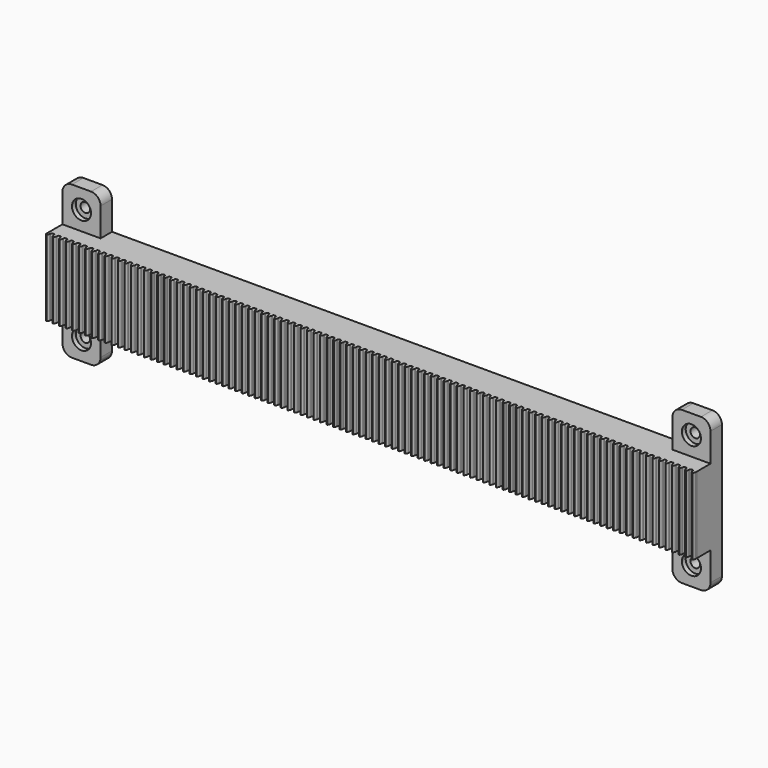
from build123d import *

# Parameters (mm, degrees)
F1_DEPTH       = 9.525
F3_D           = 6.35
F3_DEPTH       = 76.2
F3_CBORE_D     = 12.7
F3_CBORE_DEPTH = 3.175
F3_TIP         = 1.9077324654
F4_DEPTH       = 11.2014
F6_DEPTH       = 50.8


# Not quite as in the source:
# - ends of sketch curves that miss each other by under 0.0002 mm in the source are joined


with BuildPart() as f1:
    # F0 (on Front) → F1 (new body)
    with BuildSketch(Plane.XZ):
        with BuildLine():
            Line((-45.4660036325, -34.71942029), (-70.8660036325, -34.71942029))
            Line((-70.8660036325, -34.71942029), (-70.8660036325, -53.76942029))
            ThreePointArc((-70.8660036325, -53.76942029), (-69.0061316931, -58.2595483505), (-64.5160036325, -60.11942029))
            Line((-64.5160036325, -60.11942029), (-51.8160036325, -60.11942029))
            ThreePointArc((-51.8160036325, -60.11942029), (-47.325875572, -58.2595483505), (-45.4660036325, -53.76942029))
            Line((-45.4660036325, -53.76942029), (-45.4660036325, -34.71942029))
        make_face()
        with BuildLine():
            Line((360.9339963675, -34.71942029), (335.5339963675, -34.71942029))
            Line((335.5339963675, -34.71942029), (335.5339963675, -53.76942029))
            ThreePointArc((335.5339963675, -53.76942029), (337.3938683069, -58.2595483505), (341.8839963675, -60.11942029))
            Line((341.8839963675, -60.11942029), (354.5839963675, -60.11942029))
            ThreePointArc((354.5839963675, -60.11942029), (359.074124428, -58.2595483505), (360.9339963675, -53.76942029))
            Line((360.9339963675, -53.76942029), (360.9339963675, -34.71942029))
        make_face()
        with BuildLine():
            Line((-70.8660036325, 35.13057971), (-70.8660036325, 16.08057971))
            Line((-70.8660036325, 16.08057971), (-45.4660036325, 16.08057971))
            Line((-45.4660036325, 16.08057971), (-45.4660036325, 35.13057971))
            ThreePointArc((-45.4660036325, 35.13057971), (-47.325875572, 39.6207077705), (-51.8160036325, 41.48057971))
            Line((-51.8160036325, 41.48057971), (-64.5160036325, 41.48057971))
            ThreePointArc((-64.5160036325, 41.48057971), (-69.0061316931, 39.6207077705), (-70.8660036325, 35.13057971))
        make_face()
        with BuildLine():
            Line((335.5339963675, 35.13057971), (335.5339963675, 16.08057971))
            Line((335.5339963675, 16.08057971), (360.9339963675, 16.08057971))
            Line((360.9339963675, 16.08057971), (360.9339963675, 35.13057971))
            ThreePointArc((360.9339963675, 35.13057971), (359.074124428, 39.6207077705), (354.5839963675, 41.48057971))
            Line((354.5839963675, 41.48057971), (341.8839963675, 41.48057971))
            ThreePointArc((341.8839963675, 41.48057971), (337.3938683069, 39.6207077705), (335.5339963675, 35.13057971))
        make_face()
        Polygon((-70.8660036325, 16.08057971), (-70.8660036325, -34.71942029), (-45.4660036325, -34.71942029), (335.5339963675, -34.71942029), (360.9339963675, -34.71942029), (360.9339963675, 16.08057971), (335.5339963675, 16.08057971), (-45.4660036325, 16.08057971), align=None)
    extrude(amount=F1_DEPTH)

    # F3
    with Locations(Plane.XZ.offset(9.525)):
        with Locations((-58.1660036325, 28.78057971), (-58.1660036325, -47.41942029), (348.2339963675, 28.78057971), (348.2339963675, -47.41942029)):
            CounterBoreHole(F3_D / 2, F3_CBORE_D / 2, F3_CBORE_DEPTH, depth=F3_DEPTH)
            with Locations((0, 0, -(F3_DEPTH + F3_TIP / 2))):  # 118° drill point
                Cone(0, F3_D / 2, F3_TIP, mode=Mode.SUBTRACT)

    # F2 (on face) → F4 (join)
    with BuildSketch(Plane.XZ.offset(9.525)):
        Polygon((-70.8660036325, -34.71942029), (-45.4660036325, -34.71942029), (335.5339963675, -34.71942029), (360.9339963675, -34.71942029), (360.9339963675, 16.08057971), (335.5339963675, 16.08057971), (-45.4660036325, 16.08057971), (-70.8660036325, 16.08057971), align=None)
    extrude(amount=F4_DEPTH)

    # F5 (on face) → F6 (join)
    with BuildSketch(Plane.XY.offset(16.08057971)):
        with BuildLine():
            ThreePointArc((358.7730106639, -21.7934941062), (358.793978513, -22.1295298739), (358.8847933365, -22.4537402312))
            ThreePointArc((358.8847933365, -22.4537402312), (359.1204464297, -22.9793001932), (359.4003722576, -23.4826759822))
            ThreePointArc((359.4003722576, -23.4826759822), (359.5824599106, -23.6586683535), (359.8268861963, -23.7248878292))
            Line((359.8268861963, -23.7248878292), (359.8389923503, -23.7250411258))
            ThreePointArc((359.8389923503, -23.7250411258), (360.0909087908, -23.6618306043), (360.2786560778, -23.482363562))
            ThreePointArc((360.2786560778, -23.482363562), (360.5580862345, -22.9785947657), (360.7932033185, -22.4526820649))
            ThreePointArc((360.7932033185, -22.4526820649), (360.8836597236, -22.1283726389), (360.9042556369, -21.7923148461))
            Line((360.9042556369, -21.7923148461), (360.8934786021, -21.5485759988))
            ThreePointArc((360.8934786021, -21.5485759988), (360.900473163, -21.4034991932), (360.9339958063, -21.2621753247))
            Line((360.9339958063, -21.2621753247), (360.9339963675, -20.7264))
            Line((360.9339963675, -20.7264), (357.9969362179, -20.7264))
            ThreePointArc((357.9969362179, -20.7264), (358.5655750742, -20.9691454204), (358.7836056546, -21.5477110208))
            Line((358.7836056546, -21.5477110208), (358.7730106639, -21.7934941062))
        make_face()
        with BuildLine():
            ThreePointArc((356.5500786021, -21.5485759988), (356.7677699929, -20.9694547467), (357.3367100412, -20.7263946969))
            Line((357.3367100412, -20.7263946969), (356.5905959712, -20.7263946969))
            Line((356.5905959712, -20.7263946969), (353.6535362179, -20.7264))
            ThreePointArc((353.6535362179, -20.7264), (354.2221750742, -20.9691454204), (354.4402056546, -21.5477110208))
            Line((354.4402056546, -21.5477110208), (354.4296106639, -21.7934941062))
            ThreePointArc((354.4296106639, -21.7934941062), (354.450578513, -22.1295298739), (354.5413933365, -22.4537402312))
            ThreePointArc((354.5413933365, -22.4537402312), (354.7770464297, -22.9793001932), (355.0569722576, -23.4826759822))
            ThreePointArc((355.0569722576, -23.4826759822), (355.2390599106, -23.6586683535), (355.4834861963, -23.7248878292))
            Line((355.4834861963, -23.7248878292), (355.4955923503, -23.7250411258))
            ThreePointArc((355.4955923503, -23.7250411258), (355.7475087908, -23.6618306043), (355.9352560778, -23.482363562))
            ThreePointArc((355.9352560778, -23.482363562), (356.2146862345, -22.9785947657), (356.4498033185, -22.4526820649))
            ThreePointArc((356.4498033185, -22.4526820649), (356.5402597236, -22.1283726389), (356.5608556369, -21.7923148461))
            Line((356.5608556369, -21.7923148461), (356.5500786021, -21.5485759988))
        make_face()
        with BuildLine():
            ThreePointArc((352.2066786021, -21.5485759988), (352.4243699929, -20.9694547467), (352.9933100412, -20.7263946969))
            Line((352.9933100412, -20.7263946969), (352.2471959712, -20.7263946969))
            Line((352.2471959712, -20.7263946969), (349.3101362179, -20.7264))
            ThreePointArc((349.3101362179, -20.7264), (349.8787750742, -20.9691454204), (350.0968056546, -21.5477110208))
            Line((350.0968056546, -21.5477110208), (350.0862106639, -21.7934941062))
            ThreePointArc((350.0862106639, -21.7934941062), (350.107178513, -22.1295298739), (350.1979933365, -22.4537402312))
            ThreePointArc((350.1979933365, -22.4537402312), (350.4336464297, -22.9793001932), (350.7135722576, -23.4826759822))
            ThreePointArc((350.7135722576, -23.4826759822), (350.8956599106, -23.6586683535), (351.1400861963, -23.7248878292))
            Line((351.1400861963, -23.7248878292), (351.1521923503, -23.7250411258))
            ThreePointArc((351.1521923503, -23.7250411258), (351.4041087908, -23.6618306043), (351.5918560778, -23.482363562))
            ThreePointArc((351.5918560778, -23.482363562), (351.8712862345, -22.9785947657), (352.1064033185, -22.4526820649))
            ThreePointArc((352.1064033185, -22.4526820649), (352.1968597236, -22.1283726389), (352.2174556369, -21.7923148461))
            Line((352.2174556369, -21.7923148461), (352.2066786021, -21.5485759988))
        make_face()
        with BuildLine():
            ThreePointArc((347.8632786021, -21.5485759988), (348.0809699929, -20.9694547467), (348.6499100412, -20.7263946969))
            Line((348.6499100412, -20.7263946969), (347.9037959712, -20.7263946969))
            Line((347.9037959712, -20.7263946969), (344.9667362179, -20.7264))
            ThreePointArc((344.9667362179, -20.7264), (345.5353750742, -20.9691454204), (345.7534056546, -21.5477110208))
            Line((345.7534056546, -21.5477110208), (345.7428106639, -21.7934941062))
            ThreePointArc((345.7428106639, -21.7934941062), (345.763778513, -22.1295298739), (345.8545933365, -22.4537402312))
            ThreePointArc((345.8545933365, -22.4537402312), (346.0902464297, -22.9793001932), (346.3701722576, -23.4826759822))
            ThreePointArc((346.3701722576, -23.4826759822), (346.5522599106, -23.6586683535), (346.7966861963, -23.7248878292))
            Line((346.7966861963, -23.7248878292), (346.8087923503, -23.7250411258))
            ThreePointArc((346.8087923503, -23.7250411258), (347.0607087908, -23.6618306043), (347.2484560778, -23.482363562))
            ThreePointArc((347.2484560778, -23.482363562), (347.5278862345, -22.9785947657), (347.7630033185, -22.4526820649))
            ThreePointArc((347.7630033185, -22.4526820649), (347.8534597236, -22.1283726389), (347.8740556369, -21.7923148461))
            Line((347.8740556369, -21.7923148461), (347.8632786021, -21.5485759988))
        make_face()
        with BuildLine():
            ThreePointArc((343.5198786021, -21.5485759988), (343.7375699929, -20.9694547467), (344.3065100412, -20.7263946969))
            Line((344.3065100412, -20.7263946969), (343.5603959712, -20.7263946969))
            Line((343.5603959712, -20.7263946969), (340.6233362179, -20.7264))
            ThreePointArc((340.6233362179, -20.7264), (341.1919750742, -20.9691454204), (341.4100056546, -21.5477110208))
            Line((341.4100056546, -21.5477110208), (341.3994106639, -21.7934941062))
            ThreePointArc((341.3994106639, -21.7934941062), (341.420378513, -22.1295298739), (341.5111933365, -22.4537402312))
            ThreePointArc((341.5111933365, -22.4537402312), (341.7468464297, -22.9793001932), (342.0267722576, -23.4826759822))
            ThreePointArc((342.0267722576, -23.4826759822), (342.2088599106, -23.6586683535), (342.4532861963, -23.7248878292))
            Line((342.4532861963, -23.7248878292), (342.4653923503, -23.7250411258))
            ThreePointArc((342.4653923503, -23.7250411258), (342.7173087908, -23.6618306043), (342.9050560778, -23.482363562))
            ThreePointArc((342.9050560778, -23.482363562), (343.1844862345, -22.9785947657), (343.4196033185, -22.4526820649))
            ThreePointArc((343.4196033185, -22.4526820649), (343.5100597236, -22.1283726389), (343.5306556369, -21.7923148461))
            Line((343.5306556369, -21.7923148461), (343.5198786021, -21.5485759988))
        make_face()
        with BuildLine():
            ThreePointArc((339.1764786021, -21.5485759988), (339.3941699929, -20.9694547467), (339.9631100412, -20.7263946969))
            Line((339.9631100412, -20.7263946969), (339.2169959712, -20.7263946969))
            Line((339.2169959712, -20.7263946969), (336.2799362179, -20.7264))
            ThreePointArc((336.2799362179, -20.7264), (336.8485750742, -20.9691454204), (337.0666056546, -21.5477110208))
            Line((337.0666056546, -21.5477110208), (337.0560106639, -21.7934941062))
            ThreePointArc((337.0560106639, -21.7934941062), (337.076978513, -22.1295298739), (337.1677933365, -22.4537402312))
            ThreePointArc((337.1677933365, -22.4537402312), (337.4034464297, -22.9793001932), (337.6833722576, -23.4826759822))
            ThreePointArc((337.6833722576, -23.4826759822), (337.8654599106, -23.6586683535), (338.1098861963, -23.7248878292))
            Line((338.1098861963, -23.7248878292), (338.1219923503, -23.7250411258))
            ThreePointArc((338.1219923503, -23.7250411258), (338.3739087908, -23.6618306043), (338.5616560778, -23.482363562))
            ThreePointArc((338.5616560778, -23.482363562), (338.8410862345, -22.9785947657), (339.0762033185, -22.4526820649))
            ThreePointArc((339.0762033185, -22.4526820649), (339.1666597236, -22.1283726389), (339.1872556369, -21.7923148461))
            Line((339.1872556369, -21.7923148461), (339.1764786021, -21.5485759988))
        make_face()
        with BuildLine():
            ThreePointArc((334.8330786021, -21.5485759988), (335.0507699929, -20.9694547467), (335.6197100412, -20.7263946969))
            Line((335.6197100412, -20.7263946969), (334.8735959712, -20.7263946969))
            Line((334.8735959712, -20.7263946969), (331.9365362179, -20.7264))
            ThreePointArc((331.9365362179, -20.7264), (332.5051750742, -20.9691454204), (332.7232056546, -21.5477110208))
            Line((332.7232056546, -21.5477110208), (332.7126106639, -21.7934941062))
            ThreePointArc((332.7126106639, -21.7934941062), (332.733578513, -22.1295298739), (332.8243933365, -22.4537402312))
            ThreePointArc((332.8243933365, -22.4537402312), (333.0600464297, -22.9793001932), (333.3399722576, -23.4826759822))
            ThreePointArc((333.3399722576, -23.4826759822), (333.5220599106, -23.6586683535), (333.7664861963, -23.7248878292))
            Line((333.7664861963, -23.7248878292), (333.7785923503, -23.7250411258))
            ThreePointArc((333.7785923503, -23.7250411258), (334.0305087908, -23.6618306043), (334.2182560778, -23.482363562))
            ThreePointArc((334.2182560778, -23.482363562), (334.4976862345, -22.9785947657), (334.7328033185, -22.4526820649))
            ThreePointArc((334.7328033185, -22.4526820649), (334.8232597236, -22.1283726389), (334.8438556369, -21.7923148461))
            Line((334.8438556369, -21.7923148461), (334.8330786021, -21.5485759988))
        make_face()
        with BuildLine():
            ThreePointArc((330.4896786021, -21.5485759988), (330.7073699929, -20.9694547467), (331.2763100412, -20.7263946969))
            Line((331.2763100412, -20.7263946969), (330.5301959712, -20.7263946969))
            Line((330.5301959712, -20.7263946969), (327.5931362179, -20.7264))
            ThreePointArc((327.5931362179, -20.7264), (328.1617750742, -20.9691454204), (328.3798056546, -21.5477110208))
            Line((328.3798056546, -21.5477110208), (328.3692106639, -21.7934941062))
            ThreePointArc((328.3692106639, -21.7934941062), (328.390178513, -22.1295298739), (328.4809933365, -22.4537402312))
            ThreePointArc((328.4809933365, -22.4537402312), (328.7166464297, -22.9793001932), (328.9965722576, -23.4826759822))
            ThreePointArc((328.9965722576, -23.4826759822), (329.1786599106, -23.6586683535), (329.4230861963, -23.7248878292))
            Line((329.4230861963, -23.7248878292), (329.4351923503, -23.7250411258))
            ThreePointArc((329.4351923503, -23.7250411258), (329.6871087908, -23.6618306043), (329.8748560778, -23.482363562))
            ThreePointArc((329.8748560778, -23.482363562), (330.1542862345, -22.9785947657), (330.3894033185, -22.4526820649))
            ThreePointArc((330.3894033185, -22.4526820649), (330.4798597236, -22.1283726389), (330.5004556369, -21.7923148461))
            Line((330.5004556369, -21.7923148461), (330.4896786021, -21.5485759988))
        make_face()
        with BuildLine():
            ThreePointArc((326.1462786021, -21.5485759988), (326.3639699929, -20.9694547467), (326.9329100412, -20.7263946969))
            Line((326.9329100412, -20.7263946969), (326.1867959712, -20.7263946969))
            Line((326.1867959712, -20.7263946969), (323.2497362179, -20.7264))
            ThreePointArc((323.2497362179, -20.7264), (323.8183750742, -20.9691454204), (324.0364056546, -21.5477110208))
            Line((324.0364056546, -21.5477110208), (324.0258106639, -21.7934941062))
            ThreePointArc((324.0258106639, -21.7934941062), (324.046778513, -22.1295298739), (324.1375933365, -22.4537402312))
            ThreePointArc((324.1375933365, -22.4537402312), (324.3732464297, -22.9793001932), (324.6531722576, -23.4826759822))
            ThreePointArc((324.6531722576, -23.4826759822), (324.8352599106, -23.6586683535), (325.0796861963, -23.7248878292))
            Line((325.0796861963, -23.7248878292), (325.0917923503, -23.7250411258))
            ThreePointArc((325.0917923503, -23.7250411258), (325.3437087908, -23.6618306043), (325.5314560778, -23.482363562))
            ThreePointArc((325.5314560778, -23.482363562), (325.8108862345, -22.9785947657), (326.0460033185, -22.4526820649))
            ThreePointArc((326.0460033185, -22.4526820649), (326.1364597236, -22.1283726389), (326.1570556369, -21.7923148461))
            Line((326.1570556369, -21.7923148461), (326.1462786021, -21.5485759988))
        make_face()
        with BuildLine():
            ThreePointArc((321.8028786021, -21.5485759988), (322.0205699929, -20.9694547467), (322.5895100412, -20.7263946969))
            Line((322.5895100412, -20.7263946969), (321.8433959712, -20.7263946969))
            Line((321.8433959712, -20.7263946969), (318.9063362179, -20.7264))
            ThreePointArc((318.9063362179, -20.7264), (319.4749750742, -20.9691454204), (319.6930056546, -21.5477110208))
            Line((319.6930056546, -21.5477110208), (319.6824106639, -21.7934941062))
            ThreePointArc((319.6824106639, -21.7934941062), (319.703378513, -22.1295298739), (319.7941933365, -22.4537402312))
            ThreePointArc((319.7941933365, -22.4537402312), (320.0298464297, -22.9793001932), (320.3097722576, -23.4826759822))
            ThreePointArc((320.3097722576, -23.4826759822), (320.4918599106, -23.6586683535), (320.7362861963, -23.7248878292))
            Line((320.7362861963, -23.7248878292), (320.7483923503, -23.7250411258))
            ThreePointArc((320.7483923503, -23.7250411258), (321.0003087908, -23.6618306043), (321.1880560778, -23.482363562))
            ThreePointArc((321.1880560778, -23.482363562), (321.4674862345, -22.9785947657), (321.7026033185, -22.4526820649))
            ThreePointArc((321.7026033185, -22.4526820649), (321.7930597236, -22.1283726389), (321.8136556369, -21.7923148461))
            Line((321.8136556369, -21.7923148461), (321.8028786021, -21.5485759988))
        make_face()
        with BuildLine():
            ThreePointArc((317.4594786021, -21.5485759988), (317.6771699929, -20.9694547467), (318.2461100412, -20.7263946969))
            Line((318.2461100412, -20.7263946969), (317.4999959712, -20.7263946969))
            Line((317.4999959712, -20.7263946969), (314.5629362179, -20.7264))
            ThreePointArc((314.5629362179, -20.7264), (315.1315750742, -20.9691454204), (315.3496056546, -21.5477110208))
            Line((315.3496056546, -21.5477110208), (315.3390106639, -21.7934941062))
            ThreePointArc((315.3390106639, -21.7934941062), (315.359978513, -22.1295298739), (315.4507933365, -22.4537402312))
            ThreePointArc((315.4507933365, -22.4537402312), (315.6864464297, -22.9793001932), (315.9663722576, -23.4826759822))
            ThreePointArc((315.9663722576, -23.4826759822), (316.1484599106, -23.6586683535), (316.3928861963, -23.7248878292))
            Line((316.3928861963, -23.7248878292), (316.4049923503, -23.7250411258))
            ThreePointArc((316.4049923503, -23.7250411258), (316.6569087908, -23.6618306043), (316.8446560778, -23.482363562))
            ThreePointArc((316.8446560778, -23.482363562), (317.1240862345, -22.9785947657), (317.3592033185, -22.4526820649))
            ThreePointArc((317.3592033185, -22.4526820649), (317.4496597236, -22.1283726389), (317.4702556369, -21.7923148461))
            Line((317.4702556369, -21.7923148461), (317.4594786021, -21.5485759988))
        make_face()
        with BuildLine():
            ThreePointArc((313.1160786021, -21.5485759988), (313.3337699929, -20.9694547467), (313.9027100412, -20.7263946969))
            Line((313.9027100412, -20.7263946969), (313.1565959712, -20.7263946969))
            Line((313.1565959712, -20.7263946969), (310.2195362179, -20.7264))
            ThreePointArc((310.2195362179, -20.7264), (310.7881750742, -20.9691454204), (311.0062056546, -21.5477110208))
            Line((311.0062056546, -21.5477110208), (310.9956106639, -21.7934941062))
            ThreePointArc((310.9956106639, -21.7934941062), (311.016578513, -22.1295298739), (311.1073933365, -22.4537402312))
            ThreePointArc((311.1073933365, -22.4537402312), (311.3430464297, -22.9793001932), (311.6229722576, -23.4826759822))
            ThreePointArc((311.6229722576, -23.4826759822), (311.8050599106, -23.6586683535), (312.0494861963, -23.7248878292))
            Line((312.0494861963, -23.7248878292), (312.0615923503, -23.7250411258))
            ThreePointArc((312.0615923503, -23.7250411258), (312.3135087908, -23.6618306043), (312.5012560778, -23.482363562))
            ThreePointArc((312.5012560778, -23.482363562), (312.7806862345, -22.9785947657), (313.0158033185, -22.4526820649))
            ThreePointArc((313.0158033185, -22.4526820649), (313.1062597236, -22.1283726389), (313.1268556369, -21.7923148461))
            Line((313.1268556369, -21.7923148461), (313.1160786021, -21.5485759988))
        make_face()
        with BuildLine():
            ThreePointArc((308.7726786021, -21.5485759988), (308.9903699929, -20.9694547467), (309.5593100412, -20.7263946969))
            Line((309.5593100412, -20.7263946969), (308.8131959712, -20.7263946969))
            Line((308.8131959712, -20.7263946969), (305.8761362179, -20.7264))
            ThreePointArc((305.8761362179, -20.7264), (306.4447750742, -20.9691454204), (306.6628056546, -21.5477110208))
            Line((306.6628056546, -21.5477110208), (306.6522106639, -21.7934941062))
            ThreePointArc((306.6522106639, -21.7934941062), (306.673178513, -22.1295298739), (306.7639933365, -22.4537402312))
            ThreePointArc((306.7639933365, -22.4537402312), (306.9996464297, -22.9793001932), (307.2795722576, -23.4826759822))
            ThreePointArc((307.2795722576, -23.4826759822), (307.4616599106, -23.6586683535), (307.7060861963, -23.7248878292))
            Line((307.7060861963, -23.7248878292), (307.7181923503, -23.7250411258))
            ThreePointArc((307.7181923503, -23.7250411258), (307.9701087908, -23.6618306043), (308.1578560778, -23.482363562))
            ThreePointArc((308.1578560778, -23.482363562), (308.4372862345, -22.9785947657), (308.6724033185, -22.4526820649))
            ThreePointArc((308.6724033185, -22.4526820649), (308.7628597236, -22.1283726389), (308.7834556369, -21.7923148461))
            Line((308.7834556369, -21.7923148461), (308.7726786021, -21.5485759988))
        make_face()
        with BuildLine():
            ThreePointArc((304.4292786021, -21.5485759988), (304.6469699929, -20.9694547467), (305.2159100412, -20.7263946969))
            Line((305.2159100412, -20.7263946969), (304.4697959712, -20.7263946969))
            Line((304.4697959712, -20.7263946969), (301.5327362179, -20.7264))
            ThreePointArc((301.5327362179, -20.7264), (302.1013750742, -20.9691454204), (302.3194056546, -21.5477110208))
            Line((302.3194056546, -21.5477110208), (302.3088106639, -21.7934941062))
            ThreePointArc((302.3088106639, -21.7934941062), (302.329778513, -22.1295298739), (302.4205933365, -22.4537402312))
            ThreePointArc((302.4205933365, -22.4537402312), (302.6562464297, -22.9793001932), (302.9361722576, -23.4826759822))
            ThreePointArc((302.9361722576, -23.4826759822), (303.1182599106, -23.6586683535), (303.3626861963, -23.7248878292))
            Line((303.3626861963, -23.7248878292), (303.3747923503, -23.7250411258))
            ThreePointArc((303.3747923503, -23.7250411258), (303.6267087908, -23.6618306043), (303.8144560778, -23.482363562))
            ThreePointArc((303.8144560778, -23.482363562), (304.0938862345, -22.9785947657), (304.3290033185, -22.4526820649))
            ThreePointArc((304.3290033185, -22.4526820649), (304.4194597236, -22.1283726389), (304.4400556369, -21.7923148461))
            Line((304.4400556369, -21.7923148461), (304.4292786021, -21.5485759988))
        make_face()
        with BuildLine():
            ThreePointArc((300.0858786021, -21.5485759988), (300.3035699929, -20.9694547467), (300.8725100412, -20.7263946969))
            Line((300.8725100412, -20.7263946969), (300.1263959712, -20.7263946969))
            Line((300.1263959712, -20.7263946969), (297.1893362179, -20.7264))
            ThreePointArc((297.1893362179, -20.7264), (297.7579750742, -20.9691454204), (297.9760056546, -21.5477110208))
            Line((297.9760056546, -21.5477110208), (297.9654106639, -21.7934941062))
            ThreePointArc((297.9654106639, -21.7934941062), (297.986378513, -22.1295298739), (298.0771933365, -22.4537402312))
            ThreePointArc((298.0771933365, -22.4537402312), (298.3128464297, -22.9793001932), (298.5927722576, -23.4826759822))
            ThreePointArc((298.5927722576, -23.4826759822), (298.7748599106, -23.6586683535), (299.0192861963, -23.7248878292))
            Line((299.0192861963, -23.7248878292), (299.0313923503, -23.7250411258))
            ThreePointArc((299.0313923503, -23.7250411258), (299.2833087908, -23.6618306043), (299.4710560778, -23.482363562))
            ThreePointArc((299.4710560778, -23.482363562), (299.7504862345, -22.9785947657), (299.9856033185, -22.4526820649))
            ThreePointArc((299.9856033185, -22.4526820649), (300.0760597236, -22.1283726389), (300.0966556369, -21.7923148461))
            Line((300.0966556369, -21.7923148461), (300.0858786021, -21.5485759988))
        make_face()
        with BuildLine():
            ThreePointArc((295.7424786021, -21.5485759988), (295.9601699929, -20.9694547467), (296.5291100412, -20.7263946969))
            Line((296.5291100412, -20.7263946969), (295.7829959712, -20.7263946969))
            Line((295.7829959712, -20.7263946969), (292.8459362179, -20.7264))
            ThreePointArc((292.8459362179, -20.7264), (293.4145750742, -20.9691454204), (293.6326056546, -21.5477110208))
            Line((293.6326056546, -21.5477110208), (293.6220106639, -21.7934941062))
            ThreePointArc((293.6220106639, -21.7934941062), (293.642978513, -22.1295298739), (293.7337933365, -22.4537402312))
            ThreePointArc((293.7337933365, -22.4537402312), (293.9694464297, -22.9793001932), (294.2493722576, -23.4826759822))
            ThreePointArc((294.2493722576, -23.4826759822), (294.4314599106, -23.6586683535), (294.6758861963, -23.7248878292))
            Line((294.6758861963, -23.7248878292), (294.6879923503, -23.7250411258))
            ThreePointArc((294.6879923503, -23.7250411258), (294.9399087908, -23.6618306043), (295.1276560778, -23.482363562))
            ThreePointArc((295.1276560778, -23.482363562), (295.4070862345, -22.9785947657), (295.6422033185, -22.4526820649))
            ThreePointArc((295.6422033185, -22.4526820649), (295.7326597236, -22.1283726389), (295.7532556369, -21.7923148461))
            Line((295.7532556369, -21.7923148461), (295.7424786021, -21.5485759988))
        make_face()
        with BuildLine():
            ThreePointArc((291.3990786021, -21.5485759988), (291.6167699929, -20.9694547467), (292.1857100412, -20.7263946969))
            Line((292.1857100412, -20.7263946969), (291.4395959712, -20.7263946969))
            Line((291.4395959712, -20.7263946969), (288.5025362179, -20.7264))
            ThreePointArc((288.5025362179, -20.7264), (289.0711750742, -20.9691454204), (289.2892056546, -21.5477110208))
            Line((289.2892056546, -21.5477110208), (289.2786106639, -21.7934941062))
            ThreePointArc((289.2786106639, -21.7934941062), (289.299578513, -22.1295298739), (289.3903933365, -22.4537402312))
            ThreePointArc((289.3903933365, -22.4537402312), (289.6260464297, -22.9793001932), (289.9059722576, -23.4826759822))
            ThreePointArc((289.9059722576, -23.4826759822), (290.0880599106, -23.6586683535), (290.3324861963, -23.7248878292))
            Line((290.3324861963, -23.7248878292), (290.3445923503, -23.7250411258))
            ThreePointArc((290.3445923503, -23.7250411258), (290.5965087908, -23.6618306043), (290.7842560778, -23.482363562))
            ThreePointArc((290.7842560778, -23.482363562), (291.0636862345, -22.9785947657), (291.2988033185, -22.4526820649))
            ThreePointArc((291.2988033185, -22.4526820649), (291.3892597236, -22.1283726389), (291.4098556369, -21.7923148461))
            Line((291.4098556369, -21.7923148461), (291.3990786021, -21.5485759988))
        make_face()
        with BuildLine():
            ThreePointArc((287.0556786021, -21.5485759988), (287.2733699929, -20.9694547467), (287.8423100412, -20.7263946969))
            Line((287.8423100412, -20.7263946969), (287.0961959712, -20.7263946969))
            Line((287.0961959712, -20.7263946969), (284.1591362179, -20.7264))
            ThreePointArc((284.1591362179, -20.7264), (284.7277750742, -20.9691454204), (284.9458056546, -21.5477110208))
            Line((284.9458056546, -21.5477110208), (284.9352106639, -21.7934941062))
            ThreePointArc((284.9352106639, -21.7934941062), (284.956178513, -22.1295298739), (285.0469933365, -22.4537402312))
            ThreePointArc((285.0469933365, -22.4537402312), (285.2826464297, -22.9793001932), (285.5625722576, -23.4826759822))
            ThreePointArc((285.5625722576, -23.4826759822), (285.7446599106, -23.6586683535), (285.9890861963, -23.7248878292))
            Line((285.9890861963, -23.7248878292), (286.0011923503, -23.7250411258))
            ThreePointArc((286.0011923503, -23.7250411258), (286.2531087908, -23.6618306043), (286.4408560778, -23.482363562))
            ThreePointArc((286.4408560778, -23.482363562), (286.7202862345, -22.9785947657), (286.9554033185, -22.4526820649))
            ThreePointArc((286.9554033185, -22.4526820649), (287.0458597236, -22.1283726389), (287.0664556369, -21.7923148461))
            Line((287.0664556369, -21.7923148461), (287.0556786021, -21.5485759988))
        make_face()
        with BuildLine():
            ThreePointArc((282.7122786021, -21.5485759988), (282.9299699929, -20.9694547467), (283.4989100412, -20.7263946969))
            Line((283.4989100412, -20.7263946969), (282.7527959712, -20.7263946969))
            Line((282.7527959712, -20.7263946969), (279.8157362179, -20.7264))
            ThreePointArc((279.8157362179, -20.7264), (280.3843750742, -20.9691454204), (280.6024056546, -21.5477110208))
            Line((280.6024056546, -21.5477110208), (280.5918106639, -21.7934941062))
            ThreePointArc((280.5918106639, -21.7934941062), (280.612778513, -22.1295298739), (280.7035933365, -22.4537402312))
            ThreePointArc((280.7035933365, -22.4537402312), (280.9392464297, -22.9793001932), (281.2191722576, -23.4826759822))
            ThreePointArc((281.2191722576, -23.4826759822), (281.4012599106, -23.6586683535), (281.6456861963, -23.7248878292))
            Line((281.6456861963, -23.7248878292), (281.6577923503, -23.7250411258))
            ThreePointArc((281.6577923503, -23.7250411258), (281.9097087908, -23.6618306043), (282.0974560778, -23.482363562))
            ThreePointArc((282.0974560778, -23.482363562), (282.3768862345, -22.9785947657), (282.6120033185, -22.4526820649))
            ThreePointArc((282.6120033185, -22.4526820649), (282.7024597236, -22.1283726389), (282.7230556369, -21.7923148461))
            Line((282.7230556369, -21.7923148461), (282.7122786021, -21.5485759988))
        make_face()
        with BuildLine():
            ThreePointArc((278.3688786021, -21.5485759988), (278.5865699929, -20.9694547467), (279.1555100412, -20.7263946969))
            Line((279.1555100412, -20.7263946969), (278.4093959712, -20.7263946969))
            Line((278.4093959712, -20.7263946969), (275.4723362179, -20.7264))
            ThreePointArc((275.4723362179, -20.7264), (276.0409750742, -20.9691454204), (276.2590056546, -21.5477110208))
            Line((276.2590056546, -21.5477110208), (276.2484106639, -21.7934941062))
            ThreePointArc((276.2484106639, -21.7934941062), (276.269378513, -22.1295298739), (276.3601933365, -22.4537402312))
            ThreePointArc((276.3601933365, -22.4537402312), (276.5958464297, -22.9793001932), (276.8757722576, -23.4826759822))
            ThreePointArc((276.8757722576, -23.4826759822), (277.0578599106, -23.6586683535), (277.3022861963, -23.7248878292))
            Line((277.3022861963, -23.7248878292), (277.3143923503, -23.7250411258))
            ThreePointArc((277.3143923503, -23.7250411258), (277.5663087908, -23.6618306043), (277.7540560778, -23.482363562))
            ThreePointArc((277.7540560778, -23.482363562), (278.0334862345, -22.9785947657), (278.2686033185, -22.4526820649))
            ThreePointArc((278.2686033185, -22.4526820649), (278.3590597236, -22.1283726389), (278.3796556369, -21.7923148461))
            Line((278.3796556369, -21.7923148461), (278.3688786021, -21.5485759988))
        make_face()
        with BuildLine():
            ThreePointArc((274.0254786021, -21.5485759988), (274.2431699929, -20.9694547467), (274.8121100412, -20.7263946969))
            Line((274.8121100412, -20.7263946969), (274.0659959712, -20.7263946969))
            Line((274.0659959712, -20.7263946969), (271.1289362179, -20.7264))
            ThreePointArc((271.1289362179, -20.7264), (271.6975750742, -20.9691454204), (271.9156056546, -21.5477110208))
            Line((271.9156056546, -21.5477110208), (271.9050106639, -21.7934941062))
            ThreePointArc((271.9050106639, -21.7934941062), (271.925978513, -22.1295298739), (272.0167933365, -22.4537402312))
            ThreePointArc((272.0167933365, -22.4537402312), (272.2524464297, -22.9793001932), (272.5323722576, -23.4826759822))
            ThreePointArc((272.5323722576, -23.4826759822), (272.7144599106, -23.6586683535), (272.9588861963, -23.7248878292))
            Line((272.9588861963, -23.7248878292), (272.9709923503, -23.7250411258))
            ThreePointArc((272.9709923503, -23.7250411258), (273.2229087908, -23.6618306043), (273.4106560778, -23.482363562))
            ThreePointArc((273.4106560778, -23.482363562), (273.6900862345, -22.9785947657), (273.9252033185, -22.4526820649))
            ThreePointArc((273.9252033185, -22.4526820649), (274.0156597236, -22.1283726389), (274.0362556369, -21.7923148461))
            Line((274.0362556369, -21.7923148461), (274.0254786021, -21.5485759988))
        make_face()
        with BuildLine():
            ThreePointArc((269.6820786021, -21.5485759988), (269.8997699929, -20.9694547467), (270.4687100412, -20.7263946969))
            Line((270.4687100412, -20.7263946969), (269.7225959712, -20.7263946969))
            Line((269.7225959712, -20.7263946969), (266.7855362179, -20.7264))
            ThreePointArc((266.7855362179, -20.7264), (267.3541750742, -20.9691454204), (267.5722056546, -21.5477110208))
            Line((267.5722056546, -21.5477110208), (267.5616106639, -21.7934941062))
            ThreePointArc((267.5616106639, -21.7934941062), (267.582578513, -22.1295298739), (267.6733933365, -22.4537402312))
            ThreePointArc((267.6733933365, -22.4537402312), (267.9090464297, -22.9793001932), (268.1889722576, -23.4826759822))
            ThreePointArc((268.1889722576, -23.4826759822), (268.3710599106, -23.6586683535), (268.6154861963, -23.7248878292))
            Line((268.6154861963, -23.7248878292), (268.6275923503, -23.7250411258))
            ThreePointArc((268.6275923503, -23.7250411258), (268.8795087908, -23.6618306043), (269.0672560778, -23.482363562))
            ThreePointArc((269.0672560778, -23.482363562), (269.3466862345, -22.9785947657), (269.5818033185, -22.4526820649))
            ThreePointArc((269.5818033185, -22.4526820649), (269.6722597236, -22.1283726389), (269.6928556369, -21.7923148461))
            Line((269.6928556369, -21.7923148461), (269.6820786021, -21.5485759988))
        make_face()
        with BuildLine():
            ThreePointArc((265.3386786021, -21.5485759988), (265.5563699929, -20.9694547467), (266.1253100412, -20.7263946969))
            Line((266.1253100412, -20.7263946969), (265.3791959712, -20.7263946969))
            Line((265.3791959712, -20.7263946969), (262.4421362179, -20.7264))
            ThreePointArc((262.4421362179, -20.7264), (263.0107750742, -20.9691454204), (263.2288056546, -21.5477110208))
            Line((263.2288056546, -21.5477110208), (263.2182106639, -21.7934941062))
            ThreePointArc((263.2182106639, -21.7934941062), (263.239178513, -22.1295298739), (263.3299933365, -22.4537402312))
            ThreePointArc((263.3299933365, -22.4537402312), (263.5656464297, -22.9793001932), (263.8455722576, -23.4826759822))
            ThreePointArc((263.8455722576, -23.4826759822), (264.0276599106, -23.6586683535), (264.2720861963, -23.7248878292))
            Line((264.2720861963, -23.7248878292), (264.2841923503, -23.7250411258))
            ThreePointArc((264.2841923503, -23.7250411258), (264.5361087908, -23.6618306043), (264.7238560778, -23.482363562))
            ThreePointArc((264.7238560778, -23.482363562), (265.0032862345, -22.9785947657), (265.2384033185, -22.4526820649))
            ThreePointArc((265.2384033185, -22.4526820649), (265.3288597236, -22.1283726389), (265.3494556369, -21.7923148461))
            Line((265.3494556369, -21.7923148461), (265.3386786021, -21.5485759988))
        make_face()
        with BuildLine():
            ThreePointArc((260.9952786021, -21.5485759988), (261.2129699929, -20.9694547467), (261.7819100412, -20.7263946969))
            Line((261.7819100412, -20.7263946969), (261.0357959712, -20.7263946969))
            Line((261.0357959712, -20.7263946969), (258.0987362179, -20.7264))
            ThreePointArc((258.0987362179, -20.7264), (258.6673750742, -20.9691454204), (258.8854056546, -21.5477110208))
            Line((258.8854056546, -21.5477110208), (258.8748106639, -21.7934941062))
            ThreePointArc((258.8748106639, -21.7934941062), (258.895778513, -22.1295298739), (258.9865933365, -22.4537402312))
            ThreePointArc((258.9865933365, -22.4537402312), (259.2222464297, -22.9793001932), (259.5021722576, -23.4826759822))
            ThreePointArc((259.5021722576, -23.4826759822), (259.6842599106, -23.6586683535), (259.9286861963, -23.7248878292))
            Line((259.9286861963, -23.7248878292), (259.9407923503, -23.7250411258))
            ThreePointArc((259.9407923503, -23.7250411258), (260.1927087908, -23.6618306043), (260.3804560778, -23.482363562))
            ThreePointArc((260.3804560778, -23.482363562), (260.6598862345, -22.9785947657), (260.8950033185, -22.4526820649))
            ThreePointArc((260.8950033185, -22.4526820649), (260.9854597236, -22.1283726389), (261.0060556369, -21.7923148461))
            Line((261.0060556369, -21.7923148461), (260.9952786021, -21.5485759988))
        make_face()
        with BuildLine():
            ThreePointArc((256.6518786021, -21.5485759988), (256.8695699929, -20.9694547467), (257.4385100412, -20.7263946969))
            Line((257.4385100412, -20.7263946969), (256.6923959712, -20.7263946969))
            Line((256.6923959712, -20.7263946969), (253.7553362179, -20.7264))
            ThreePointArc((253.7553362179, -20.7264), (254.3239750742, -20.9691454204), (254.5420056546, -21.5477110208))
            Line((254.5420056546, -21.5477110208), (254.5314106639, -21.7934941062))
            ThreePointArc((254.5314106639, -21.7934941062), (254.552378513, -22.1295298739), (254.6431933365, -22.4537402312))
            ThreePointArc((254.6431933365, -22.4537402312), (254.8788464297, -22.9793001932), (255.1587722576, -23.4826759822))
            ThreePointArc((255.1587722576, -23.4826759822), (255.3408599106, -23.6586683535), (255.5852861963, -23.7248878292))
            Line((255.5852861963, -23.7248878292), (255.5973923503, -23.7250411258))
            ThreePointArc((255.5973923503, -23.7250411258), (255.8493087908, -23.6618306043), (256.0370560778, -23.482363562))
            ThreePointArc((256.0370560778, -23.482363562), (256.3164862345, -22.9785947657), (256.5516033185, -22.4526820649))
            ThreePointArc((256.5516033185, -22.4526820649), (256.6420597236, -22.1283726389), (256.6626556369, -21.7923148461))
            Line((256.6626556369, -21.7923148461), (256.6518786021, -21.5485759988))
        make_face()
        with BuildLine():
            ThreePointArc((252.3084786021, -21.5485759988), (252.5261699929, -20.9694547467), (253.0951100412, -20.7263946969))
            Line((253.0951100412, -20.7263946969), (252.3489959712, -20.7263946969))
            Line((252.3489959712, -20.7263946969), (249.4119362179, -20.7264))
            ThreePointArc((249.4119362179, -20.7264), (249.9805750742, -20.9691454204), (250.1986056546, -21.5477110208))
            Line((250.1986056546, -21.5477110208), (250.1880106639, -21.7934941062))
            ThreePointArc((250.1880106639, -21.7934941062), (250.208978513, -22.1295298739), (250.2997933365, -22.4537402312))
            ThreePointArc((250.2997933365, -22.4537402312), (250.5354464297, -22.9793001932), (250.8153722576, -23.4826759822))
            ThreePointArc((250.8153722576, -23.4826759822), (250.9974599106, -23.6586683535), (251.2418861963, -23.7248878292))
            Line((251.2418861963, -23.7248878292), (251.2539923503, -23.7250411258))
            ThreePointArc((251.2539923503, -23.7250411258), (251.5059087908, -23.6618306043), (251.6936560778, -23.482363562))
            ThreePointArc((251.6936560778, -23.482363562), (251.9730862345, -22.9785947657), (252.2082033185, -22.4526820649))
            ThreePointArc((252.2082033185, -22.4526820649), (252.2986597236, -22.1283726389), (252.3192556369, -21.7923148461))
            Line((252.3192556369, -21.7923148461), (252.3084786021, -21.5485759988))
        make_face()
        with BuildLine():
            ThreePointArc((247.9650786021, -21.5485759988), (248.1827699929, -20.9694547467), (248.7517100412, -20.7263946969))
            Line((248.7517100412, -20.7263946969), (248.0055959712, -20.7263946969))
            Line((248.0055959712, -20.7263946969), (245.0685362179, -20.7264))
            ThreePointArc((245.0685362179, -20.7264), (245.6371750742, -20.9691454204), (245.8552056546, -21.5477110208))
            Line((245.8552056546, -21.5477110208), (245.8446106639, -21.7934941062))
            ThreePointArc((245.8446106639, -21.7934941062), (245.865578513, -22.1295298739), (245.9563933365, -22.4537402312))
            ThreePointArc((245.9563933365, -22.4537402312), (246.1920464297, -22.9793001932), (246.4719722576, -23.4826759822))
            ThreePointArc((246.4719722576, -23.4826759822), (246.6540599106, -23.6586683535), (246.8984861963, -23.7248878292))
            Line((246.8984861963, -23.7248878292), (246.9105923503, -23.7250411258))
            ThreePointArc((246.9105923503, -23.7250411258), (247.1625087908, -23.6618306043), (247.3502560778, -23.482363562))
            ThreePointArc((247.3502560778, -23.482363562), (247.6296862345, -22.9785947657), (247.8648033185, -22.4526820649))
            ThreePointArc((247.8648033185, -22.4526820649), (247.9552597236, -22.1283726389), (247.9758556369, -21.7923148461))
            Line((247.9758556369, -21.7923148461), (247.9650786021, -21.5485759988))
        make_face()
        with BuildLine():
            ThreePointArc((243.6216786021, -21.5485759988), (243.8393699929, -20.9694547467), (244.4083100412, -20.7263946969))
            Line((244.4083100412, -20.7263946969), (243.6621959712, -20.7263946969))
            Line((243.6621959712, -20.7263946969), (240.7251362179, -20.7264))
            ThreePointArc((240.7251362179, -20.7264), (241.2937750742, -20.9691454204), (241.5118056546, -21.5477110208))
            Line((241.5118056546, -21.5477110208), (241.5012106639, -21.7934941062))
            ThreePointArc((241.5012106639, -21.7934941062), (241.522178513, -22.1295298739), (241.6129933365, -22.4537402312))
            ThreePointArc((241.6129933365, -22.4537402312), (241.8486464297, -22.9793001932), (242.1285722576, -23.4826759822))
            ThreePointArc((242.1285722576, -23.4826759822), (242.3106599106, -23.6586683535), (242.5550861963, -23.7248878292))
            Line((242.5550861963, -23.7248878292), (242.5671923503, -23.7250411258))
            ThreePointArc((242.5671923503, -23.7250411258), (242.8191087908, -23.6618306043), (243.0068560778, -23.482363562))
            ThreePointArc((243.0068560778, -23.482363562), (243.2862862345, -22.9785947657), (243.5214033185, -22.4526820649))
            ThreePointArc((243.5214033185, -22.4526820649), (243.6118597236, -22.1283726389), (243.6324556369, -21.7923148461))
            Line((243.6324556369, -21.7923148461), (243.6216786021, -21.5485759988))
        make_face()
        with BuildLine():
            ThreePointArc((239.2782786021, -21.5485759988), (239.4959699929, -20.9694547467), (240.0649100412, -20.7263946969))
            Line((240.0649100412, -20.7263946969), (239.3187959712, -20.7263946969))
            Line((239.3187959712, -20.7263946969), (236.3817362179, -20.7264))
            ThreePointArc((236.3817362179, -20.7264), (236.9503750742, -20.9691454204), (237.1684056546, -21.5477110208))
            Line((237.1684056546, -21.5477110208), (237.1578106639, -21.7934941062))
            ThreePointArc((237.1578106639, -21.7934941062), (237.178778513, -22.1295298739), (237.2695933365, -22.4537402312))
            ThreePointArc((237.2695933365, -22.4537402312), (237.5052464297, -22.9793001932), (237.7851722576, -23.4826759822))
            ThreePointArc((237.7851722576, -23.4826759822), (237.9672599106, -23.6586683535), (238.2116861963, -23.7248878292))
            Line((238.2116861963, -23.7248878292), (238.2237923503, -23.7250411258))
            ThreePointArc((238.2237923503, -23.7250411258), (238.4757087908, -23.6618306043), (238.6634560778, -23.482363562))
            ThreePointArc((238.6634560778, -23.482363562), (238.9428862345, -22.9785947657), (239.1780033185, -22.4526820649))
            ThreePointArc((239.1780033185, -22.4526820649), (239.2684597236, -22.1283726389), (239.2890556369, -21.7923148461))
            Line((239.2890556369, -21.7923148461), (239.2782786021, -21.5485759988))
        make_face()
        with BuildLine():
            ThreePointArc((234.9348786021, -21.5485759988), (235.1525699929, -20.9694547467), (235.7215100412, -20.7263946969))
            Line((235.7215100412, -20.7263946969), (234.9753959712, -20.7263946969))
            Line((234.9753959712, -20.7263946969), (232.0383362179, -20.7264))
            ThreePointArc((232.0383362179, -20.7264), (232.6069750742, -20.9691454204), (232.8250056546, -21.5477110208))
            Line((232.8250056546, -21.5477110208), (232.8144106639, -21.7934941062))
            ThreePointArc((232.8144106639, -21.7934941062), (232.835378513, -22.1295298739), (232.9261933365, -22.4537402312))
            ThreePointArc((232.9261933365, -22.4537402312), (233.1618464297, -22.9793001932), (233.4417722576, -23.4826759822))
            ThreePointArc((233.4417722576, -23.4826759822), (233.6238599106, -23.6586683535), (233.8682861963, -23.7248878292))
            Line((233.8682861963, -23.7248878292), (233.8803923503, -23.7250411258))
            ThreePointArc((233.8803923503, -23.7250411258), (234.1323087908, -23.6618306043), (234.3200560778, -23.482363562))
            ThreePointArc((234.3200560778, -23.482363562), (234.5994862345, -22.9785947657), (234.8346033185, -22.4526820649))
            ThreePointArc((234.8346033185, -22.4526820649), (234.9250597236, -22.1283726389), (234.9456556369, -21.7923148461))
            Line((234.9456556369, -21.7923148461), (234.9348786021, -21.5485759988))
        make_face()
        with BuildLine():
            ThreePointArc((230.5914786021, -21.5485759988), (230.8091699929, -20.9694547467), (231.3781100412, -20.7263946969))
            Line((231.3781100412, -20.7263946969), (230.6319959712, -20.7263946969))
            Line((230.6319959712, -20.7263946969), (227.6949362179, -20.7264))
            ThreePointArc((227.6949362179, -20.7264), (228.2635750742, -20.9691454204), (228.4816056546, -21.5477110208))
            Line((228.4816056546, -21.5477110208), (228.4710106639, -21.7934941062))
            ThreePointArc((228.4710106639, -21.7934941062), (228.491978513, -22.1295298739), (228.5827933365, -22.4537402312))
            ThreePointArc((228.5827933365, -22.4537402312), (228.8184464297, -22.9793001932), (229.0983722576, -23.4826759822))
            ThreePointArc((229.0983722576, -23.4826759822), (229.2804599106, -23.6586683535), (229.5248861963, -23.7248878292))
            Line((229.5248861963, -23.7248878292), (229.5369923503, -23.7250411258))
            ThreePointArc((229.5369923503, -23.7250411258), (229.7889087908, -23.6618306043), (229.9766560778, -23.482363562))
            ThreePointArc((229.9766560778, -23.482363562), (230.2560862345, -22.9785947657), (230.4912033185, -22.4526820649))
            ThreePointArc((230.4912033185, -22.4526820649), (230.5816597236, -22.1283726389), (230.6022556369, -21.7923148461))
            Line((230.6022556369, -21.7923148461), (230.5914786021, -21.5485759988))
        make_face()
        with BuildLine():
            ThreePointArc((226.2480786021, -21.5485759988), (226.4657699929, -20.9694547467), (227.0347100412, -20.7263946969))
            Line((227.0347100412, -20.7263946969), (226.2885959712, -20.7263946969))
            Line((226.2885959712, -20.7263946969), (223.3515362179, -20.7264))
            ThreePointArc((223.3515362179, -20.7264), (223.9201750742, -20.9691454204), (224.1382056546, -21.5477110208))
            Line((224.1382056546, -21.5477110208), (224.1276106639, -21.7934941062))
            ThreePointArc((224.1276106639, -21.7934941062), (224.148578513, -22.1295298739), (224.2393933365, -22.4537402312))
            ThreePointArc((224.2393933365, -22.4537402312), (224.4750464297, -22.9793001932), (224.7549722576, -23.4826759822))
            ThreePointArc((224.7549722576, -23.4826759822), (224.9370599106, -23.6586683535), (225.1814861963, -23.7248878292))
            Line((225.1814861963, -23.7248878292), (225.1935923503, -23.7250411258))
            ThreePointArc((225.1935923503, -23.7250411258), (225.4455087908, -23.6618306043), (225.6332560778, -23.482363562))
            ThreePointArc((225.6332560778, -23.482363562), (225.9126862345, -22.9785947657), (226.1478033185, -22.4526820649))
            ThreePointArc((226.1478033185, -22.4526820649), (226.2382597236, -22.1283726389), (226.2588556369, -21.7923148461))
            Line((226.2588556369, -21.7923148461), (226.2480786021, -21.5485759988))
        make_face()
        with BuildLine():
            ThreePointArc((221.9046786021, -21.5485759988), (222.1223699929, -20.9694547467), (222.6913100412, -20.7263946969))
            Line((222.6913100412, -20.7263946969), (221.9451959712, -20.7263946969))
            Line((221.9451959712, -20.7263946969), (219.0081362179, -20.7264))
            ThreePointArc((219.0081362179, -20.7264), (219.5767750742, -20.9691454204), (219.7948056546, -21.5477110208))
            Line((219.7948056546, -21.5477110208), (219.7842106639, -21.7934941062))
            ThreePointArc((219.7842106639, -21.7934941062), (219.805178513, -22.1295298739), (219.8959933365, -22.4537402312))
            ThreePointArc((219.8959933365, -22.4537402312), (220.1316464297, -22.9793001932), (220.4115722576, -23.4826759822))
            ThreePointArc((220.4115722576, -23.4826759822), (220.5936599106, -23.6586683535), (220.8380861963, -23.7248878292))
            Line((220.8380861963, -23.7248878292), (220.8501923503, -23.7250411258))
            ThreePointArc((220.8501923503, -23.7250411258), (221.1021087908, -23.6618306043), (221.2898560778, -23.482363562))
            ThreePointArc((221.2898560778, -23.482363562), (221.5692862345, -22.9785947657), (221.8044033185, -22.4526820649))
            ThreePointArc((221.8044033185, -22.4526820649), (221.8948597236, -22.1283726389), (221.9154556369, -21.7923148461))
            Line((221.9154556369, -21.7923148461), (221.9046786021, -21.5485759988))
        make_face()
        with BuildLine():
            ThreePointArc((217.5612786021, -21.5485759988), (217.7789699929, -20.9694547467), (218.3479100412, -20.7263946969))
            Line((218.3479100412, -20.7263946969), (217.6017959712, -20.7263946969))
            Line((217.6017959712, -20.7263946969), (214.6647362179, -20.7264))
            ThreePointArc((214.6647362179, -20.7264), (215.2333750742, -20.9691454204), (215.4514056546, -21.5477110208))
            Line((215.4514056546, -21.5477110208), (215.4408106639, -21.7934941062))
            ThreePointArc((215.4408106639, -21.7934941062), (215.461778513, -22.1295298739), (215.5525933365, -22.4537402312))
            ThreePointArc((215.5525933365, -22.4537402312), (215.7882464297, -22.9793001932), (216.0681722576, -23.4826759822))
            ThreePointArc((216.0681722576, -23.4826759822), (216.2502599106, -23.6586683535), (216.4946861963, -23.7248878292))
            Line((216.4946861963, -23.7248878292), (216.5067923503, -23.7250411258))
            ThreePointArc((216.5067923503, -23.7250411258), (216.7587087908, -23.6618306043), (216.9464560778, -23.482363562))
            ThreePointArc((216.9464560778, -23.482363562), (217.2258862345, -22.9785947657), (217.4610033185, -22.4526820649))
            ThreePointArc((217.4610033185, -22.4526820649), (217.5514597236, -22.1283726389), (217.5720556369, -21.7923148461))
            Line((217.5720556369, -21.7923148461), (217.5612786021, -21.5485759988))
        make_face()
        with BuildLine():
            ThreePointArc((213.2178786021, -21.5485759988), (213.4355699929, -20.9694547467), (214.0045100412, -20.7263946969))
            Line((214.0045100412, -20.7263946969), (213.2583959712, -20.7263946969))
            Line((213.2583959712, -20.7263946969), (210.3213362179, -20.7264))
            ThreePointArc((210.3213362179, -20.7264), (210.8899750742, -20.9691454204), (211.1080056546, -21.5477110208))
            Line((211.1080056546, -21.5477110208), (211.0974106639, -21.7934941062))
            ThreePointArc((211.0974106639, -21.7934941062), (211.118378513, -22.1295298739), (211.2091933365, -22.4537402312))
            ThreePointArc((211.2091933365, -22.4537402312), (211.4448464297, -22.9793001932), (211.7247722576, -23.4826759822))
            ThreePointArc((211.7247722576, -23.4826759822), (211.9068599106, -23.6586683535), (212.1512861963, -23.7248878292))
            Line((212.1512861963, -23.7248878292), (212.1633923503, -23.7250411258))
            ThreePointArc((212.1633923503, -23.7250411258), (212.4153087908, -23.6618306043), (212.6030560778, -23.482363562))
            ThreePointArc((212.6030560778, -23.482363562), (212.8824862345, -22.9785947657), (213.1176033185, -22.4526820649))
            ThreePointArc((213.1176033185, -22.4526820649), (213.2080597236, -22.1283726389), (213.2286556369, -21.7923148461))
            Line((213.2286556369, -21.7923148461), (213.2178786021, -21.5485759988))
        make_face()
        with BuildLine():
            ThreePointArc((191.5008786021, -21.5485759988), (191.7185699929, -20.9694547467), (192.2875100412, -20.7263946969))
            Line((192.2875100412, -20.7263946969), (191.5413959712, -20.7263946969))
            Line((191.5413959712, -20.7263946969), (188.6043362179, -20.7264))
            ThreePointArc((188.6043362179, -20.7264), (189.1729750742, -20.9691454204), (189.3910056546, -21.5477110208))
            Line((189.3910056546, -21.5477110208), (189.3804106639, -21.7934941062))
            ThreePointArc((189.3804106639, -21.7934941062), (189.401378513, -22.1295298739), (189.4921933365, -22.4537402312))
            ThreePointArc((189.4921933365, -22.4537402312), (189.7278464297, -22.9793001932), (190.0077722576, -23.4826759822))
            ThreePointArc((190.0077722576, -23.4826759822), (190.1898599106, -23.6586683535), (190.4342861963, -23.7248878292))
            Line((190.4342861963, -23.7248878292), (190.4463923503, -23.7250411258))
            ThreePointArc((190.4463923503, -23.7250411258), (190.6983087908, -23.6618306043), (190.8860560778, -23.482363562))
            ThreePointArc((190.8860560778, -23.482363562), (191.1654862345, -22.9785947657), (191.4006033185, -22.4526820649))
            ThreePointArc((191.4006033185, -22.4526820649), (191.4910597236, -22.1283726389), (191.5116556369, -21.7923148461))
            Line((191.5116556369, -21.7923148461), (191.5008786021, -21.5485759988))
        make_face()
        with BuildLine():
            ThreePointArc((187.1574786021, -21.5485759988), (187.3751699929, -20.9694547467), (187.9441100412, -20.7263946969))
            Line((187.9441100412, -20.7263946969), (187.1979959712, -20.7263946969))
            Line((187.1979959712, -20.7263946969), (184.2609362179, -20.7264))
            ThreePointArc((184.2609362179, -20.7264), (184.8295750742, -20.9691454204), (185.0476056546, -21.5477110208))
            Line((185.0476056546, -21.5477110208), (185.0370106639, -21.7934941062))
            ThreePointArc((185.0370106639, -21.7934941062), (185.057978513, -22.1295298739), (185.1487933365, -22.4537402312))
            ThreePointArc((185.1487933365, -22.4537402312), (185.3844464297, -22.9793001932), (185.6643722576, -23.4826759822))
            ThreePointArc((185.6643722576, -23.4826759822), (185.8464599106, -23.6586683535), (186.0908861963, -23.7248878292))
            Line((186.0908861963, -23.7248878292), (186.1029923503, -23.7250411258))
            ThreePointArc((186.1029923503, -23.7250411258), (186.3549087908, -23.6618306043), (186.5426560778, -23.482363562))
            ThreePointArc((186.5426560778, -23.482363562), (186.8220862345, -22.9785947657), (187.0572033185, -22.4526820649))
            ThreePointArc((187.0572033185, -22.4526820649), (187.1476597236, -22.1283726389), (187.1682556369, -21.7923148461))
            Line((187.1682556369, -21.7923148461), (187.1574786021, -21.5485759988))
        make_face()
        with BuildLine():
            ThreePointArc((182.8140786021, -21.5485759988), (183.0317699929, -20.9694547467), (183.6007100412, -20.7263946969))
            Line((183.6007100412, -20.7263946969), (182.8545959712, -20.7263946969))
            Line((182.8545959712, -20.7263946969), (179.9175362179, -20.7264))
            ThreePointArc((179.9175362179, -20.7264), (180.4861750742, -20.9691454204), (180.7042056546, -21.5477110208))
            Line((180.7042056546, -21.5477110208), (180.6936106639, -21.7934941062))
            ThreePointArc((180.6936106639, -21.7934941062), (180.714578513, -22.1295298739), (180.8053933365, -22.4537402312))
            ThreePointArc((180.8053933365, -22.4537402312), (181.0410464297, -22.9793001932), (181.3209722576, -23.4826759822))
            ThreePointArc((181.3209722576, -23.4826759822), (181.5030599106, -23.6586683535), (181.7474861963, -23.7248878292))
            Line((181.7474861963, -23.7248878292), (181.7595923503, -23.7250411258))
            ThreePointArc((181.7595923503, -23.7250411258), (182.0115087908, -23.6618306043), (182.1992560778, -23.482363562))
            ThreePointArc((182.1992560778, -23.482363562), (182.4786862345, -22.9785947657), (182.7138033185, -22.4526820649))
            ThreePointArc((182.7138033185, -22.4526820649), (182.8042597236, -22.1283726389), (182.8248556369, -21.7923148461))
            Line((182.8248556369, -21.7923148461), (182.8140786021, -21.5485759988))
        make_face()
        with BuildLine():
            ThreePointArc((178.4706786021, -21.5485759988), (178.6883699929, -20.9694547467), (179.2573100412, -20.7263946969))
            Line((179.2573100412, -20.7263946969), (178.5111959712, -20.7263946969))
            Line((178.5111959712, -20.7263946969), (175.5741362179, -20.7264))
            ThreePointArc((175.5741362179, -20.7264), (176.1427750742, -20.9691454204), (176.3608056546, -21.5477110208))
            Line((176.3608056546, -21.5477110208), (176.3502106639, -21.7934941062))
            ThreePointArc((176.3502106639, -21.7934941062), (176.371178513, -22.1295298739), (176.4619933365, -22.4537402312))
            ThreePointArc((176.4619933365, -22.4537402312), (176.6976464297, -22.9793001932), (176.9775722576, -23.4826759822))
            ThreePointArc((176.9775722576, -23.4826759822), (177.1596599106, -23.6586683535), (177.4040861963, -23.7248878292))
            Line((177.4040861963, -23.7248878292), (177.4161923503, -23.7250411258))
            ThreePointArc((177.4161923503, -23.7250411258), (177.6681087908, -23.6618306043), (177.8558560778, -23.482363562))
            ThreePointArc((177.8558560778, -23.482363562), (178.1352862345, -22.9785947657), (178.3704033185, -22.4526820649))
            ThreePointArc((178.3704033185, -22.4526820649), (178.4608597236, -22.1283726389), (178.4814556369, -21.7923148461))
            Line((178.4814556369, -21.7923148461), (178.4706786021, -21.5485759988))
        make_face()
        with BuildLine():
            ThreePointArc((174.1272786021, -21.5485759988), (174.3449699929, -20.9694547467), (174.9139100412, -20.7263946969))
            Line((174.9139100412, -20.7263946969), (174.1677959712, -20.7263946969))
            Line((174.1677959712, -20.7263946969), (171.2307362179, -20.7264))
            ThreePointArc((171.2307362179, -20.7264), (171.7993750742, -20.9691454204), (172.0174056546, -21.5477110208))
            Line((172.0174056546, -21.5477110208), (172.0068106639, -21.7934941062))
            ThreePointArc((172.0068106639, -21.7934941062), (172.027778513, -22.1295298739), (172.1185933365, -22.4537402312))
            ThreePointArc((172.1185933365, -22.4537402312), (172.3542464297, -22.9793001932), (172.6341722576, -23.4826759822))
            ThreePointArc((172.6341722576, -23.4826759822), (172.8162599106, -23.6586683535), (173.0606861963, -23.7248878292))
            Line((173.0606861963, -23.7248878292), (173.0727923503, -23.7250411258))
            ThreePointArc((173.0727923503, -23.7250411258), (173.3247087908, -23.6618306043), (173.5124560778, -23.482363562))
            ThreePointArc((173.5124560778, -23.482363562), (173.7918862345, -22.9785947657), (174.0270033185, -22.4526820649))
            ThreePointArc((174.0270033185, -22.4526820649), (174.1174597236, -22.1283726389), (174.1380556369, -21.7923148461))
            Line((174.1380556369, -21.7923148461), (174.1272786021, -21.5485759988))
        make_face()
        with BuildLine():
            ThreePointArc((169.7838786021, -21.5485759988), (170.0015699929, -20.9694547467), (170.5705100412, -20.7263946969))
            Line((170.5705100412, -20.7263946969), (169.8243959712, -20.7263946969))
            Line((169.8243959712, -20.7263946969), (166.8873362179, -20.7264))
            ThreePointArc((166.8873362179, -20.7264), (167.4559750742, -20.9691454204), (167.6740056546, -21.5477110208))
            Line((167.6740056546, -21.5477110208), (167.6634106639, -21.7934941062))
            ThreePointArc((167.6634106639, -21.7934941062), (167.684378513, -22.1295298739), (167.7751933365, -22.4537402312))
            ThreePointArc((167.7751933365, -22.4537402312), (168.0108464297, -22.9793001932), (168.2907722576, -23.4826759822))
            ThreePointArc((168.2907722576, -23.4826759822), (168.4728599106, -23.6586683535), (168.7172861963, -23.7248878292))
            Line((168.7172861963, -23.7248878292), (168.7293923503, -23.7250411258))
            ThreePointArc((168.7293923503, -23.7250411258), (168.9813087908, -23.6618306043), (169.1690560778, -23.482363562))
            ThreePointArc((169.1690560778, -23.482363562), (169.4484862345, -22.9785947657), (169.6836033185, -22.4526820649))
            ThreePointArc((169.6836033185, -22.4526820649), (169.7740597236, -22.1283726389), (169.7946556369, -21.7923148461))
            Line((169.7946556369, -21.7923148461), (169.7838786021, -21.5485759988))
        make_face()
        with BuildLine():
            ThreePointArc((165.4404786021, -21.5485759988), (165.6581699929, -20.9694547467), (166.2271100412, -20.7263946969))
            Line((166.2271100412, -20.7263946969), (165.4809959712, -20.7263946969))
            Line((165.4809959712, -20.7263946969), (162.5439362179, -20.7264))
            ThreePointArc((162.5439362179, -20.7264), (163.1125750742, -20.9691454204), (163.3306056546, -21.5477110208))
            Line((163.3306056546, -21.5477110208), (163.3200106639, -21.7934941062))
            ThreePointArc((163.3200106639, -21.7934941062), (163.340978513, -22.1295298739), (163.4317933365, -22.4537402312))
            ThreePointArc((163.4317933365, -22.4537402312), (163.6674464297, -22.9793001932), (163.9473722576, -23.4826759822))
            ThreePointArc((163.9473722576, -23.4826759822), (164.1294599106, -23.6586683535), (164.3738861963, -23.7248878292))
            Line((164.3738861963, -23.7248878292), (164.3859923503, -23.7250411258))
            ThreePointArc((164.3859923503, -23.7250411258), (164.6379087908, -23.6618306043), (164.8256560778, -23.482363562))
            ThreePointArc((164.8256560778, -23.482363562), (165.1050862345, -22.9785947657), (165.3402033185, -22.4526820649))
            ThreePointArc((165.3402033185, -22.4526820649), (165.4306597236, -22.1283726389), (165.4512556369, -21.7923148461))
            Line((165.4512556369, -21.7923148461), (165.4404786021, -21.5485759988))
        make_face()
        with BuildLine():
            ThreePointArc((161.0970786021, -21.5485759988), (161.3147699929, -20.9694547467), (161.8837100412, -20.7263946969))
            Line((161.8837100412, -20.7263946969), (161.1375959712, -20.7263946969))
            Line((161.1375959712, -20.7263946969), (158.2005362179, -20.7264))
            ThreePointArc((158.2005362179, -20.7264), (158.7691750742, -20.9691454204), (158.9872056546, -21.5477110208))
            Line((158.9872056546, -21.5477110208), (158.9766106639, -21.7934941062))
            ThreePointArc((158.9766106639, -21.7934941062), (158.997578513, -22.1295298739), (159.0883933365, -22.4537402312))
            ThreePointArc((159.0883933365, -22.4537402312), (159.3240464297, -22.9793001932), (159.6039722576, -23.4826759822))
            ThreePointArc((159.6039722576, -23.4826759822), (159.7860599106, -23.6586683535), (160.0304861963, -23.7248878292))
            Line((160.0304861963, -23.7248878292), (160.0425923503, -23.7250411258))
            ThreePointArc((160.0425923503, -23.7250411258), (160.2945087908, -23.6618306043), (160.4822560778, -23.482363562))
            ThreePointArc((160.4822560778, -23.482363562), (160.7616862345, -22.9785947657), (160.9968033185, -22.4526820649))
            ThreePointArc((160.9968033185, -22.4526820649), (161.0872597236, -22.1283726389), (161.1078556369, -21.7923148461))
            Line((161.1078556369, -21.7923148461), (161.0970786021, -21.5485759988))
        make_face()
        with BuildLine():
            ThreePointArc((156.7536786021, -21.5485759988), (156.9713699929, -20.9694547467), (157.5403100412, -20.7263946969))
            Line((157.5403100412, -20.7263946969), (156.7941959712, -20.7263946969))
            Line((156.7941959712, -20.7263946969), (153.8571362179, -20.7264))
            ThreePointArc((153.8571362179, -20.7264), (154.4257750742, -20.9691454204), (154.6438056546, -21.5477110208))
            Line((154.6438056546, -21.5477110208), (154.6332106639, -21.7934941062))
            ThreePointArc((154.6332106639, -21.7934941062), (154.654178513, -22.1295298739), (154.7449933365, -22.4537402312))
            ThreePointArc((154.7449933365, -22.4537402312), (154.9806464297, -22.9793001932), (155.2605722576, -23.4826759822))
            ThreePointArc((155.2605722576, -23.4826759822), (155.4426599106, -23.6586683535), (155.6870861963, -23.7248878292))
            Line((155.6870861963, -23.7248878292), (155.6991923503, -23.7250411258))
            ThreePointArc((155.6991923503, -23.7250411258), (155.9511087908, -23.6618306043), (156.1388560778, -23.482363562))
            ThreePointArc((156.1388560778, -23.482363562), (156.4182862345, -22.9785947657), (156.6534033185, -22.4526820649))
            ThreePointArc((156.6534033185, -22.4526820649), (156.7438597236, -22.1283726389), (156.7644556369, -21.7923148461))
            Line((156.7644556369, -21.7923148461), (156.7536786021, -21.5485759988))
        make_face()
        with BuildLine():
            ThreePointArc((152.4102786021, -21.5485759988), (152.6279699929, -20.9694547467), (153.1969100412, -20.7263946969))
            Line((153.1969100412, -20.7263946969), (152.4507959712, -20.7263946969))
            Line((152.4507959712, -20.7263946969), (149.5137362179, -20.7264))
            ThreePointArc((149.5137362179, -20.7264), (150.0823750742, -20.9691454204), (150.3004056546, -21.5477110208))
            Line((150.3004056546, -21.5477110208), (150.2898106639, -21.7934941062))
            ThreePointArc((150.2898106639, -21.7934941062), (150.310778513, -22.1295298739), (150.4015933365, -22.4537402312))
            ThreePointArc((150.4015933365, -22.4537402312), (150.6372464297, -22.9793001932), (150.9171722576, -23.4826759822))
            ThreePointArc((150.9171722576, -23.4826759822), (151.0992599106, -23.6586683535), (151.3436861963, -23.7248878292))
            Line((151.3436861963, -23.7248878292), (151.3557923503, -23.7250411258))
            ThreePointArc((151.3557923503, -23.7250411258), (151.6077087908, -23.6618306043), (151.7954560778, -23.482363562))
            ThreePointArc((151.7954560778, -23.482363562), (152.0748862345, -22.9785947657), (152.3100033185, -22.4526820649))
            ThreePointArc((152.3100033185, -22.4526820649), (152.4004597236, -22.1283726389), (152.4210556369, -21.7923148461))
            Line((152.4210556369, -21.7923148461), (152.4102786021, -21.5485759988))
        make_face()
        with BuildLine():
            ThreePointArc((148.0668786021, -21.5485759988), (148.2845699929, -20.9694547467), (148.8535100412, -20.7263946969))
            Line((148.8535100412, -20.7263946969), (148.1073959712, -20.7263946969))
            Line((148.1073959712, -20.7263946969), (145.1703362179, -20.7264))
            ThreePointArc((145.1703362179, -20.7264), (145.7389750742, -20.9691454204), (145.9570056546, -21.5477110208))
            Line((145.9570056546, -21.5477110208), (145.9464106639, -21.7934941062))
            ThreePointArc((145.9464106639, -21.7934941062), (145.967378513, -22.1295298739), (146.0581933365, -22.4537402312))
            ThreePointArc((146.0581933365, -22.4537402312), (146.2938464297, -22.9793001932), (146.5737722576, -23.4826759822))
            ThreePointArc((146.5737722576, -23.4826759822), (146.7558599106, -23.6586683535), (147.0002861963, -23.7248878292))
            Line((147.0002861963, -23.7248878292), (147.0123923503, -23.7250411258))
            ThreePointArc((147.0123923503, -23.7250411258), (147.2643087908, -23.6618306043), (147.4520560778, -23.482363562))
            ThreePointArc((147.4520560778, -23.482363562), (147.7314862345, -22.9785947657), (147.9666033185, -22.4526820649))
            ThreePointArc((147.9666033185, -22.4526820649), (148.0570597236, -22.1283726389), (148.0776556369, -21.7923148461))
            Line((148.0776556369, -21.7923148461), (148.0668786021, -21.5485759988))
        make_face()
        with BuildLine():
            ThreePointArc((143.7234786021, -21.5485759988), (143.9411699929, -20.9694547467), (144.5101100412, -20.7263946969))
            Line((144.5101100412, -20.7263946969), (143.7639959712, -20.7263946969))
            Line((143.7639959712, -20.7263946969), (140.8269362179, -20.7264))
            ThreePointArc((140.8269362179, -20.7264), (141.3955750742, -20.9691454204), (141.6136056546, -21.5477110208))
            Line((141.6136056546, -21.5477110208), (141.6030106639, -21.7934941062))
            ThreePointArc((141.6030106639, -21.7934941062), (141.623978513, -22.1295298739), (141.7147933365, -22.4537402312))
            ThreePointArc((141.7147933365, -22.4537402312), (141.9504464297, -22.9793001932), (142.2303722576, -23.4826759822))
            ThreePointArc((142.2303722576, -23.4826759822), (142.4124599106, -23.6586683535), (142.6568861963, -23.7248878292))
            Line((142.6568861963, -23.7248878292), (142.6689923503, -23.7250411258))
            ThreePointArc((142.6689923503, -23.7250411258), (142.9209087908, -23.6618306043), (143.1086560778, -23.482363562))
            ThreePointArc((143.1086560778, -23.482363562), (143.3880862345, -22.9785947657), (143.6232033185, -22.4526820649))
            ThreePointArc((143.6232033185, -22.4526820649), (143.7136597236, -22.1283726389), (143.7342556369, -21.7923148461))
            Line((143.7342556369, -21.7923148461), (143.7234786021, -21.5485759988))
        make_face()
        with BuildLine():
            ThreePointArc((208.8744786021, -21.5485759988), (209.0921699929, -20.9694547467), (209.6611100412, -20.7263946969))
            Line((209.6611100412, -20.7263946969), (208.9149959712, -20.7263946969))
            Line((208.9149959712, -20.7263946969), (205.9779362179, -20.7264))
            ThreePointArc((205.9779362179, -20.7264), (206.5465750742, -20.9691454204), (206.7646056546, -21.5477110208))
            Line((206.7646056546, -21.5477110208), (206.7540106639, -21.7934941062))
            ThreePointArc((206.7540106639, -21.7934941062), (206.774978513, -22.1295298739), (206.8657933365, -22.4537402312))
            ThreePointArc((206.8657933365, -22.4537402312), (207.1014464297, -22.9793001932), (207.3813722576, -23.4826759822))
            ThreePointArc((207.3813722576, -23.4826759822), (207.5634599106, -23.6586683535), (207.8078861963, -23.7248878292))
            Line((207.8078861963, -23.7248878292), (207.8199923503, -23.7250411258))
            ThreePointArc((207.8199923503, -23.7250411258), (208.0719087908, -23.6618306043), (208.2596560778, -23.482363562))
            ThreePointArc((208.2596560778, -23.482363562), (208.5390862345, -22.9785947657), (208.7742033185, -22.4526820649))
            ThreePointArc((208.7742033185, -22.4526820649), (208.8646597236, -22.1283726389), (208.8852556369, -21.7923148461))
            Line((208.8852556369, -21.7923148461), (208.8744786021, -21.5485759988))
        make_face()
        with BuildLine():
            ThreePointArc((204.5310786021, -21.5485759988), (204.7487699929, -20.9694547467), (205.3177100412, -20.7263946969))
            Line((205.3177100412, -20.7263946969), (204.5715959712, -20.7263946969))
            Line((204.5715959712, -20.7263946969), (201.6345362179, -20.7264))
            ThreePointArc((201.6345362179, -20.7264), (202.2031750742, -20.9691454204), (202.4212056546, -21.5477110208))
            Line((202.4212056546, -21.5477110208), (202.4106106639, -21.7934941062))
            ThreePointArc((202.4106106639, -21.7934941062), (202.431578513, -22.1295298739), (202.5223933365, -22.4537402312))
            ThreePointArc((202.5223933365, -22.4537402312), (202.7580464297, -22.9793001932), (203.0379722576, -23.4826759822))
            ThreePointArc((203.0379722576, -23.4826759822), (203.2200599106, -23.6586683535), (203.4644861963, -23.7248878292))
            Line((203.4644861963, -23.7248878292), (203.4765923503, -23.7250411258))
            ThreePointArc((203.4765923503, -23.7250411258), (203.7285087908, -23.6618306043), (203.9162560778, -23.482363562))
            ThreePointArc((203.9162560778, -23.482363562), (204.1956862345, -22.9785947657), (204.4308033185, -22.4526820649))
            ThreePointArc((204.4308033185, -22.4526820649), (204.5212597236, -22.1283726389), (204.5418556369, -21.7923148461))
            Line((204.5418556369, -21.7923148461), (204.5310786021, -21.5485759988))
        make_face()
        with BuildLine():
            ThreePointArc((200.1876786021, -21.5485759988), (200.4053699929, -20.9694547467), (200.9743100412, -20.7263946969))
            Line((200.9743100412, -20.7263946969), (200.2281959712, -20.7263946969))
            Line((200.2281959712, -20.7263946969), (197.2911362179, -20.7264))
            ThreePointArc((197.2911362179, -20.7264), (197.8597750742, -20.9691454204), (198.0778056546, -21.5477110208))
            Line((198.0778056546, -21.5477110208), (198.0672106639, -21.7934941062))
            ThreePointArc((198.0672106639, -21.7934941062), (198.088178513, -22.1295298739), (198.1789933365, -22.4537402312))
            ThreePointArc((198.1789933365, -22.4537402312), (198.4146464297, -22.9793001932), (198.6945722576, -23.4826759822))
            ThreePointArc((198.6945722576, -23.4826759822), (198.8766599106, -23.6586683535), (199.1210861963, -23.7248878292))
            Line((199.1210861963, -23.7248878292), (199.1331923503, -23.7250411258))
            ThreePointArc((199.1331923503, -23.7250411258), (199.3851087908, -23.6618306043), (199.5728560778, -23.482363562))
            ThreePointArc((199.5728560778, -23.482363562), (199.8522862345, -22.9785947657), (200.0874033185, -22.4526820649))
            ThreePointArc((200.0874033185, -22.4526820649), (200.1778597236, -22.1283726389), (200.1984556369, -21.7923148461))
            Line((200.1984556369, -21.7923148461), (200.1876786021, -21.5485759988))
        make_face()
        with BuildLine():
            ThreePointArc((195.8442786021, -21.5485759988), (196.0619699929, -20.9694547467), (196.6309100412, -20.7263946969))
            Line((196.6309100412, -20.7263946969), (195.8847959712, -20.7263946969))
            Line((195.8847959712, -20.7263946969), (192.9477362179, -20.7264))
            ThreePointArc((192.9477362179, -20.7264), (193.5163750742, -20.9691454204), (193.7344056546, -21.5477110208))
            Line((193.7344056546, -21.5477110208), (193.7238106639, -21.7934941062))
            ThreePointArc((193.7238106639, -21.7934941062), (193.744778513, -22.1295298739), (193.8355933365, -22.4537402312))
            ThreePointArc((193.8355933365, -22.4537402312), (194.0712464297, -22.9793001932), (194.3511722576, -23.4826759822))
            ThreePointArc((194.3511722576, -23.4826759822), (194.5332599106, -23.6586683535), (194.7776861963, -23.7248878292))
            Line((194.7776861963, -23.7248878292), (194.7897923503, -23.7250411258))
            ThreePointArc((194.7897923503, -23.7250411258), (195.0417087908, -23.6618306043), (195.2294560778, -23.482363562))
            ThreePointArc((195.2294560778, -23.482363562), (195.5088862345, -22.9785947657), (195.7440033185, -22.4526820649))
            ThreePointArc((195.7440033185, -22.4526820649), (195.8344597236, -22.1283726389), (195.8550556369, -21.7923148461))
            Line((195.8550556369, -21.7923148461), (195.8442786021, -21.5485759988))
        make_face()
        with BuildLine():
            ThreePointArc((139.3800786021, -21.5485759988), (139.5977699929, -20.9694547467), (140.1667100412, -20.7263946969))
            Line((140.1667100412, -20.7263946969), (139.4205959712, -20.7263946969))
            Line((139.4205959712, -20.7263946969), (136.4835362179, -20.7264))
            ThreePointArc((136.4835362179, -20.7264), (137.0521750742, -20.9691454204), (137.2702056546, -21.5477110208))
            Line((137.2702056546, -21.5477110208), (137.2596106639, -21.7934941062))
            ThreePointArc((137.2596106639, -21.7934941062), (137.280578513, -22.1295298739), (137.3713933365, -22.4537402312))
            ThreePointArc((137.3713933365, -22.4537402312), (137.6070464297, -22.9793001932), (137.8869722576, -23.4826759822))
            ThreePointArc((137.8869722576, -23.4826759822), (138.0690599106, -23.6586683535), (138.3134861963, -23.7248878292))
            Line((138.3134861963, -23.7248878292), (138.3255923503, -23.7250411258))
            ThreePointArc((138.3255923503, -23.7250411258), (138.5775087908, -23.6618306043), (138.7652560778, -23.482363562))
            ThreePointArc((138.7652560778, -23.482363562), (139.0446862345, -22.9785947657), (139.2798033185, -22.4526820649))
            ThreePointArc((139.2798033185, -22.4526820649), (139.3702597236, -22.1283726389), (139.3908556369, -21.7923148461))
            Line((139.3908556369, -21.7923148461), (139.3800786021, -21.5485759988))
        make_face()
        with BuildLine():
            Line((135.0771959712, -20.7264), (132.1401362179, -20.7264))
            ThreePointArc((132.1401362179, -20.7264), (132.7087750742, -20.9691454204), (132.9268056546, -21.5477110208))
            Line((132.9268056546, -21.5477110208), (132.9162106639, -21.7934941062))
            ThreePointArc((132.9162106639, -21.7934941062), (132.937178513, -22.1295298739), (133.0279933365, -22.4537402312))
            ThreePointArc((133.0279933365, -22.4537402312), (133.2636464297, -22.9793001932), (133.5435722576, -23.4826759822))
            ThreePointArc((133.5435722576, -23.4826759822), (133.7256599106, -23.6586683535), (133.9700861963, -23.7248878292))
            Line((133.9700861963, -23.7248878292), (133.9821923503, -23.7250411258))
            ThreePointArc((133.9821923503, -23.7250411258), (134.2341087908, -23.6618306043), (134.4218560778, -23.482363562))
            ThreePointArc((134.4218560778, -23.482363562), (134.7012862345, -22.9785947657), (134.9364033185, -22.4526820649))
            ThreePointArc((134.9364033185, -22.4526820649), (135.0268597236, -22.1283726389), (135.0474556369, -21.7923148461))
            Line((135.0474556369, -21.7923148461), (135.0366786021, -21.5485759988))
            ThreePointArc((135.0366786021, -21.5485759988), (135.2543699929, -20.9694547467), (135.8233100412, -20.7263946969))
            Line((135.8233100412, -20.7263946969), (135.0771959712, -20.7264))
        make_face()
        with BuildLine():
            Line((130.7337959712, -20.7264), (127.7967362179, -20.7264))
            ThreePointArc((127.7967362179, -20.7264), (128.3653750742, -20.9691454204), (128.5834056546, -21.5477110208))
            Line((128.5834056546, -21.5477110208), (128.5728106639, -21.7934941062))
            ThreePointArc((128.5728106639, -21.7934941062), (128.593778513, -22.1295298739), (128.6845933365, -22.4537402312))
            ThreePointArc((128.6845933365, -22.4537402312), (128.9202464297, -22.9793001932), (129.2001722576, -23.4826759822))
            ThreePointArc((129.2001722576, -23.4826759822), (129.3822599106, -23.6586683535), (129.6266861963, -23.7248878292))
            Line((129.6266861963, -23.7248878292), (129.6387923503, -23.7250411258))
            ThreePointArc((129.6387923503, -23.7250411258), (129.8907087908, -23.6618306043), (130.0784560778, -23.482363562))
            ThreePointArc((130.0784560778, -23.482363562), (130.3578862345, -22.9785947657), (130.5930033185, -22.4526820649))
            ThreePointArc((130.5930033185, -22.4526820649), (130.6834597236, -22.1283726389), (130.7040556369, -21.7923148461))
            Line((130.7040556369, -21.7923148461), (130.6932786021, -21.5485759988))
            ThreePointArc((130.6932786021, -21.5485759988), (130.9109699929, -20.9694547467), (131.4799100412, -20.7263946969))
            Line((131.4799100412, -20.7263946969), (130.7337959712, -20.7264))
        make_face()
        with BuildLine():
            Line((126.3903959712, -20.7264), (123.4533362179, -20.7264))
            ThreePointArc((123.4533362179, -20.7264), (124.0219750742, -20.9691454204), (124.2400056546, -21.5477110208))
            Line((124.2400056546, -21.5477110208), (124.2294106639, -21.7934941062))
            ThreePointArc((124.2294106639, -21.7934941062), (124.250378513, -22.1295298739), (124.3411933365, -22.4537402312))
            ThreePointArc((124.3411933365, -22.4537402312), (124.5768464297, -22.9793001932), (124.8567722576, -23.4826759822))
            ThreePointArc((124.8567722576, -23.4826759822), (125.0388599106, -23.6586683535), (125.2832861963, -23.7248878292))
            Line((125.2832861963, -23.7248878292), (125.2953923503, -23.7250411258))
            ThreePointArc((125.2953923503, -23.7250411258), (125.5473087908, -23.6618306043), (125.7350560778, -23.482363562))
            ThreePointArc((125.7350560778, -23.482363562), (126.0144862345, -22.9785947657), (126.2496033185, -22.4526820649))
            ThreePointArc((126.2496033185, -22.4526820649), (126.3400597236, -22.1283726389), (126.3606556369, -21.7923148461))
            Line((126.3606556369, -21.7923148461), (126.3498786021, -21.5485759988))
            ThreePointArc((126.3498786021, -21.5485759988), (126.5675699929, -20.9694547467), (127.1365100412, -20.7263946969))
            Line((127.1365100412, -20.7263946969), (126.3903959712, -20.7264))
        make_face()
        with BuildLine():
            Line((122.0469959712, -20.7264), (119.1099362179, -20.7264))
            ThreePointArc((119.1099362179, -20.7264), (119.6785750742, -20.9691454204), (119.8966056546, -21.5477110208))
            Line((119.8966056546, -21.5477110208), (119.8860106639, -21.7934941062))
            ThreePointArc((119.8860106639, -21.7934941062), (119.906978513, -22.1295298739), (119.9977933365, -22.4537402312))
            ThreePointArc((119.9977933365, -22.4537402312), (120.2334464297, -22.9793001932), (120.5133722576, -23.4826759822))
            ThreePointArc((120.5133722576, -23.4826759822), (120.6954599106, -23.6586683535), (120.9398861963, -23.7248878292))
            Line((120.9398861963, -23.7248878292), (120.9519923503, -23.7250411258))
            ThreePointArc((120.9519923503, -23.7250411258), (121.2039087908, -23.6618306043), (121.3916560778, -23.482363562))
            ThreePointArc((121.3916560778, -23.482363562), (121.6710862345, -22.9785947657), (121.9062033185, -22.4526820649))
            ThreePointArc((121.9062033185, -22.4526820649), (121.9966597236, -22.1283726389), (122.0172556369, -21.7923148461))
            Line((122.0172556369, -21.7923148461), (122.0064786021, -21.5485759988))
            ThreePointArc((122.0064786021, -21.5485759988), (122.2241699929, -20.9694547467), (122.7931100412, -20.7263946969))
            Line((122.7931100412, -20.7263946969), (122.0469959712, -20.7264))
        make_face()
        with BuildLine():
            Line((117.7035959712, -20.7264), (114.7665362179, -20.7264))
            ThreePointArc((114.7665362179, -20.7264), (115.3351750742, -20.9691454204), (115.5532056546, -21.5477110208))
            Line((115.5532056546, -21.5477110208), (115.5426106639, -21.7934941062))
            ThreePointArc((115.5426106639, -21.7934941062), (115.563578513, -22.1295298739), (115.6543933365, -22.4537402312))
            ThreePointArc((115.6543933365, -22.4537402312), (115.8900464297, -22.9793001932), (116.1699722576, -23.4826759822))
            ThreePointArc((116.1699722576, -23.4826759822), (116.3520599106, -23.6586683535), (116.5964861963, -23.7248878292))
            Line((116.5964861963, -23.7248878292), (116.6085923503, -23.7250411258))
            ThreePointArc((116.6085923503, -23.7250411258), (116.8605087908, -23.6618306043), (117.0482560778, -23.482363562))
            ThreePointArc((117.0482560778, -23.482363562), (117.3276862345, -22.9785947657), (117.5628033185, -22.4526820649))
            ThreePointArc((117.5628033185, -22.4526820649), (117.6532597236, -22.1283726389), (117.6738556369, -21.7923148461))
            Line((117.6738556369, -21.7923148461), (117.6630786021, -21.5485759988))
            ThreePointArc((117.6630786021, -21.5485759988), (117.8807699929, -20.9694547467), (118.4497100412, -20.7263946969))
            Line((118.4497100412, -20.7263946969), (117.7035959712, -20.7264))
        make_face()
        with BuildLine():
            Line((113.3601959712, -20.7264), (110.4231362179, -20.7264))
            ThreePointArc((110.4231362179, -20.7264), (110.9917750742, -20.9691454204), (111.2098056546, -21.5477110208))
            Line((111.2098056546, -21.5477110208), (111.1992106639, -21.7934941062))
            ThreePointArc((111.1992106639, -21.7934941062), (111.220178513, -22.1295298739), (111.3109933365, -22.4537402312))
            ThreePointArc((111.3109933365, -22.4537402312), (111.5466464297, -22.9793001932), (111.8265722576, -23.4826759822))
            ThreePointArc((111.8265722576, -23.4826759822), (112.0086599106, -23.6586683535), (112.2530861963, -23.7248878292))
            Line((112.2530861963, -23.7248878292), (112.2651923503, -23.7250411258))
            ThreePointArc((112.2651923503, -23.7250411258), (112.5171087908, -23.6618306043), (112.7048560778, -23.482363562))
            ThreePointArc((112.7048560778, -23.482363562), (112.9842862345, -22.9785947657), (113.2194033185, -22.4526820649))
            ThreePointArc((113.2194033185, -22.4526820649), (113.3098597236, -22.1283726389), (113.3304556369, -21.7923148461))
            Line((113.3304556369, -21.7923148461), (113.3196786021, -21.5485759988))
            ThreePointArc((113.3196786021, -21.5485759988), (113.5373699929, -20.9694547467), (114.1063100412, -20.7263946969))
            Line((114.1063100412, -20.7263946969), (113.3601959712, -20.7264))
        make_face()
        with BuildLine():
            Line((109.0167959712, -20.7264), (106.0797362179, -20.7264))
            ThreePointArc((106.0797362179, -20.7264), (106.6483750742, -20.9691454204), (106.8664056546, -21.5477110208))
            Line((106.8664056546, -21.5477110208), (106.8558106639, -21.7934941062))
            ThreePointArc((106.8558106639, -21.7934941062), (106.876778513, -22.1295298739), (106.9675933365, -22.4537402312))
            ThreePointArc((106.9675933365, -22.4537402312), (107.2032464297, -22.9793001932), (107.4831722576, -23.4826759822))
            ThreePointArc((107.4831722576, -23.4826759822), (107.6652599106, -23.6586683535), (107.9096861963, -23.7248878292))
            Line((107.9096861963, -23.7248878292), (107.9217923503, -23.7250411258))
            ThreePointArc((107.9217923503, -23.7250411258), (108.1737087908, -23.6618306043), (108.3614560778, -23.482363562))
            ThreePointArc((108.3614560778, -23.482363562), (108.6408862345, -22.9785947657), (108.8760033185, -22.4526820649))
            ThreePointArc((108.8760033185, -22.4526820649), (108.9664597236, -22.1283726389), (108.9870556369, -21.7923148461))
            Line((108.9870556369, -21.7923148461), (108.9762786021, -21.5485759988))
            ThreePointArc((108.9762786021, -21.5485759988), (109.1939699929, -20.9694547467), (109.7629100412, -20.7263946969))
            Line((109.7629100412, -20.7263946969), (109.0167959712, -20.7264))
        make_face()
        with BuildLine():
            Line((104.6733959712, -20.7264), (101.7363362179, -20.7264))
            ThreePointArc((101.7363362179, -20.7264), (102.3049750742, -20.9691454204), (102.5230056546, -21.5477110208))
            Line((102.5230056546, -21.5477110208), (102.5124106639, -21.7934941062))
            ThreePointArc((102.5124106639, -21.7934941062), (102.533378513, -22.1295298739), (102.6241933365, -22.4537402312))
            ThreePointArc((102.6241933365, -22.4537402312), (102.8598464297, -22.9793001932), (103.1397722576, -23.4826759822))
            ThreePointArc((103.1397722576, -23.4826759822), (103.3218599106, -23.6586683535), (103.5662861963, -23.7248878292))
            Line((103.5662861963, -23.7248878292), (103.5783923503, -23.7250411258))
            ThreePointArc((103.5783923503, -23.7250411258), (103.8303087908, -23.6618306043), (104.0180560778, -23.482363562))
            ThreePointArc((104.0180560778, -23.482363562), (104.2974862345, -22.9785947657), (104.5326033185, -22.4526820649))
            ThreePointArc((104.5326033185, -22.4526820649), (104.6230597236, -22.1283726389), (104.6436556369, -21.7923148461))
            Line((104.6436556369, -21.7923148461), (104.6328786021, -21.5485759988))
            ThreePointArc((104.6328786021, -21.5485759988), (104.8505699929, -20.9694547467), (105.4195100412, -20.7263946969))
            Line((105.4195100412, -20.7263946969), (104.6733959712, -20.7264))
        make_face()
        with BuildLine():
            Line((100.3299959712, -20.7264), (97.3929362179, -20.7264))
            ThreePointArc((97.3929362179, -20.7264), (97.9615750742, -20.9691454204), (98.1796056546, -21.5477110208))
            Line((98.1796056546, -21.5477110208), (98.1690106639, -21.7934941062))
            ThreePointArc((98.1690106639, -21.7934941062), (98.189978513, -22.1295298739), (98.2807933365, -22.4537402312))
            ThreePointArc((98.2807933365, -22.4537402312), (98.5164464297, -22.9793001932), (98.7963722576, -23.4826759822))
            ThreePointArc((98.7963722576, -23.4826759822), (98.9784599106, -23.6586683535), (99.2228861963, -23.7248878292))
            Line((99.2228861963, -23.7248878292), (99.2349923503, -23.7250411258))
            ThreePointArc((99.2349923503, -23.7250411258), (99.4869087908, -23.6618306043), (99.6746560778, -23.482363562))
            ThreePointArc((99.6746560778, -23.482363562), (99.9540862345, -22.9785947657), (100.1892033185, -22.4526820649))
            ThreePointArc((100.1892033185, -22.4526820649), (100.2796597236, -22.1283726389), (100.3002556369, -21.7923148461))
            Line((100.3002556369, -21.7923148461), (100.2894786021, -21.5485759988))
            ThreePointArc((100.2894786021, -21.5485759988), (100.5071699929, -20.9694547467), (101.0761100412, -20.7263946969))
            Line((101.0761100412, -20.7263946969), (100.3299959712, -20.7264))
        make_face()
        with BuildLine():
            Line((95.9865959712, -20.7264), (93.0495362179, -20.7264))
            ThreePointArc((93.0495362179, -20.7264), (93.6181750742, -20.9691454204), (93.8362056546, -21.5477110208))
            Line((93.8362056546, -21.5477110208), (93.8256106639, -21.7934941062))
            ThreePointArc((93.8256106639, -21.7934941062), (93.846578513, -22.1295298739), (93.9373933365, -22.4537402312))
            ThreePointArc((93.9373933365, -22.4537402312), (94.1730464297, -22.9793001932), (94.4529722576, -23.4826759822))
            ThreePointArc((94.4529722576, -23.4826759822), (94.6350599106, -23.6586683535), (94.8794861963, -23.7248878292))
            Line((94.8794861963, -23.7248878292), (94.8915923503, -23.7250411258))
            ThreePointArc((94.8915923503, -23.7250411258), (95.1435087908, -23.6618306043), (95.3312560778, -23.482363562))
            ThreePointArc((95.3312560778, -23.482363562), (95.6106862345, -22.9785947657), (95.8458033185, -22.4526820649))
            ThreePointArc((95.8458033185, -22.4526820649), (95.9362597236, -22.1283726389), (95.9568556369, -21.7923148461))
            Line((95.9568556369, -21.7923148461), (95.9460786021, -21.5485759988))
            ThreePointArc((95.9460786021, -21.5485759988), (96.1637699929, -20.9694547467), (96.7327100412, -20.7263946969))
            Line((96.7327100412, -20.7263946969), (95.9865959712, -20.7264))
        make_face()
        with BuildLine():
            Line((91.6431959712, -20.7264), (88.7061362179, -20.7264))
            ThreePointArc((88.7061362179, -20.7264), (89.2747750742, -20.9691454204), (89.4928056546, -21.5477110208))
            Line((89.4928056546, -21.5477110208), (89.4822106639, -21.7934941062))
            ThreePointArc((89.4822106639, -21.7934941062), (89.503178513, -22.1295298739), (89.5939933365, -22.4537402312))
            ThreePointArc((89.5939933365, -22.4537402312), (89.8296464297, -22.9793001932), (90.1095722576, -23.4826759822))
            ThreePointArc((90.1095722576, -23.4826759822), (90.2916599106, -23.6586683535), (90.5360861963, -23.7248878292))
            Line((90.5360861963, -23.7248878292), (90.5481923503, -23.7250411258))
            ThreePointArc((90.5481923503, -23.7250411258), (90.8001087908, -23.6618306043), (90.9878560778, -23.482363562))
            ThreePointArc((90.9878560778, -23.482363562), (91.2672862345, -22.9785947657), (91.5024033185, -22.4526820649))
            ThreePointArc((91.5024033185, -22.4526820649), (91.5928597236, -22.1283726389), (91.6134556369, -21.7923148461))
            Line((91.6134556369, -21.7923148461), (91.6026786021, -21.5485759988))
            ThreePointArc((91.6026786021, -21.5485759988), (91.8203699929, -20.9694547467), (92.3893100412, -20.7263946969))
            Line((92.3893100412, -20.7263946969), (91.6431959712, -20.7264))
        make_face()
        with BuildLine():
            Line((87.2997959712, -20.7264), (84.3627362179, -20.7264))
            ThreePointArc((84.3627362179, -20.7264), (84.9313750742, -20.9691454204), (85.1494056546, -21.5477110208))
            Line((85.1494056546, -21.5477110208), (85.1388106639, -21.7934941062))
            ThreePointArc((85.1388106639, -21.7934941062), (85.159778513, -22.1295298739), (85.2505933365, -22.4537402312))
            ThreePointArc((85.2505933365, -22.4537402312), (85.4862464297, -22.9793001932), (85.7661722576, -23.4826759822))
            ThreePointArc((85.7661722576, -23.4826759822), (85.9482599106, -23.6586683535), (86.1926861963, -23.7248878292))
            Line((86.1926861963, -23.7248878292), (86.2047923503, -23.7250411258))
            ThreePointArc((86.2047923503, -23.7250411258), (86.4567087908, -23.6618306043), (86.6444560778, -23.482363562))
            ThreePointArc((86.6444560778, -23.482363562), (86.9238862345, -22.9785947657), (87.1590033185, -22.4526820649))
            ThreePointArc((87.1590033185, -22.4526820649), (87.2494597236, -22.1283726389), (87.2700556369, -21.7923148461))
            Line((87.2700556369, -21.7923148461), (87.2592786021, -21.5485759988))
            ThreePointArc((87.2592786021, -21.5485759988), (87.4769699929, -20.9694547467), (88.0459100412, -20.7263946969))
            Line((88.0459100412, -20.7263946969), (87.2997959712, -20.7264))
        make_face()
        with BuildLine():
            Line((82.9563959712, -20.7264), (80.0193362179, -20.7264))
            ThreePointArc((80.0193362179, -20.7264), (80.5879750742, -20.9691454204), (80.8060056546, -21.5477110208))
            Line((80.8060056546, -21.5477110208), (80.7954106639, -21.7934941062))
            ThreePointArc((80.7954106639, -21.7934941062), (80.816378513, -22.1295298739), (80.9071933365, -22.4537402312))
            ThreePointArc((80.9071933365, -22.4537402312), (81.1428464297, -22.9793001932), (81.4227722576, -23.4826759822))
            ThreePointArc((81.4227722576, -23.4826759822), (81.6048599106, -23.6586683535), (81.8492861963, -23.7248878292))
            Line((81.8492861963, -23.7248878292), (81.8613923503, -23.7250411258))
            ThreePointArc((81.8613923503, -23.7250411258), (82.1133087908, -23.6618306043), (82.3010560778, -23.482363562))
            ThreePointArc((82.3010560778, -23.482363562), (82.5804862345, -22.9785947657), (82.8156033185, -22.4526820649))
            ThreePointArc((82.8156033185, -22.4526820649), (82.9060597236, -22.1283726389), (82.9266556369, -21.7923148461))
            Line((82.9266556369, -21.7923148461), (82.9158786021, -21.5485759988))
            ThreePointArc((82.9158786021, -21.5485759988), (83.1335699929, -20.9694547467), (83.7025100412, -20.7263946969))
            Line((83.7025100412, -20.7263946969), (82.9563959712, -20.7264))
        make_face()
        with BuildLine():
            Line((78.6129959712, -20.7264), (75.6759362179, -20.7264))
            ThreePointArc((75.6759362179, -20.7264), (76.2445750742, -20.9691454204), (76.4626056546, -21.5477110208))
            Line((76.4626056546, -21.5477110208), (76.4520106639, -21.7934941062))
            ThreePointArc((76.4520106639, -21.7934941062), (76.472978513, -22.1295298739), (76.5637933365, -22.4537402312))
            ThreePointArc((76.5637933365, -22.4537402312), (76.7994464297, -22.9793001932), (77.0793722576, -23.4826759822))
            ThreePointArc((77.0793722576, -23.4826759822), (77.2614599106, -23.6586683535), (77.5058861963, -23.7248878292))
            Line((77.5058861963, -23.7248878292), (77.5179923503, -23.7250411258))
            ThreePointArc((77.5179923503, -23.7250411258), (77.7699087908, -23.6618306043), (77.9576560778, -23.482363562))
            ThreePointArc((77.9576560778, -23.482363562), (78.2370862345, -22.9785947657), (78.4722033185, -22.4526820649))
            ThreePointArc((78.4722033185, -22.4526820649), (78.5626597236, -22.1283726389), (78.5832556369, -21.7923148461))
            Line((78.5832556369, -21.7923148461), (78.5724786021, -21.5485759988))
            ThreePointArc((78.5724786021, -21.5485759988), (78.7901699929, -20.9694547467), (79.3591100412, -20.7263946969))
            Line((79.3591100412, -20.7263946969), (78.6129959712, -20.7264))
        make_face()
        with BuildLine():
            Line((74.2695959712, -20.7264), (71.3325362179, -20.7264))
            ThreePointArc((71.3325362179, -20.7264), (71.9011750742, -20.9691454204), (72.1192056546, -21.5477110208))
            Line((72.1192056546, -21.5477110208), (72.1086106639, -21.7934941062))
            ThreePointArc((72.1086106639, -21.7934941062), (72.129578513, -22.1295298739), (72.2203933365, -22.4537402312))
            ThreePointArc((72.2203933365, -22.4537402312), (72.4560464297, -22.9793001932), (72.7359722576, -23.4826759822))
            ThreePointArc((72.7359722576, -23.4826759822), (72.9180599106, -23.6586683535), (73.1624861963, -23.7248878292))
            Line((73.1624861963, -23.7248878292), (73.1745923503, -23.7250411258))
            ThreePointArc((73.1745923503, -23.7250411258), (73.4265087908, -23.6618306043), (73.6142560778, -23.482363562))
            ThreePointArc((73.6142560778, -23.482363562), (73.8936862345, -22.9785947657), (74.1288033185, -22.4526820649))
            ThreePointArc((74.1288033185, -22.4526820649), (74.2192597236, -22.1283726389), (74.2398556369, -21.7923148461))
            Line((74.2398556369, -21.7923148461), (74.2290786021, -21.5485759988))
            ThreePointArc((74.2290786021, -21.5485759988), (74.4467699929, -20.9694547467), (75.0157100412, -20.7263946969))
            Line((75.0157100412, -20.7263946969), (74.2695959712, -20.7264))
        make_face()
        with BuildLine():
            Line((69.9261959712, -20.7264), (66.9891362179, -20.7264))
            ThreePointArc((66.9891362179, -20.7264), (67.5577750742, -20.9691454204), (67.7758056546, -21.5477110208))
            Line((67.7758056546, -21.5477110208), (67.7652106639, -21.7934941062))
            ThreePointArc((67.7652106639, -21.7934941062), (67.786178513, -22.1295298739), (67.8769933365, -22.4537402312))
            ThreePointArc((67.8769933365, -22.4537402312), (68.1126464297, -22.9793001932), (68.3925722576, -23.4826759822))
            ThreePointArc((68.3925722576, -23.4826759822), (68.5746599106, -23.6586683535), (68.8190861963, -23.7248878292))
            Line((68.8190861963, -23.7248878292), (68.8311923503, -23.7250411258))
            ThreePointArc((68.8311923503, -23.7250411258), (69.0831087908, -23.6618306043), (69.2708560778, -23.482363562))
            ThreePointArc((69.2708560778, -23.482363562), (69.5502862345, -22.9785947657), (69.7854033185, -22.4526820649))
            ThreePointArc((69.7854033185, -22.4526820649), (69.8758597236, -22.1283726389), (69.8964556369, -21.7923148461))
            Line((69.8964556369, -21.7923148461), (69.8856786021, -21.5485759988))
            ThreePointArc((69.8856786021, -21.5485759988), (70.1033699929, -20.9694547467), (70.6723100412, -20.7263946969))
            Line((70.6723100412, -20.7263946969), (69.9261959712, -20.7264))
        make_face()
        with BuildLine():
            Line((65.5827959712, -20.7264), (62.6457362179, -20.7264))
            ThreePointArc((62.6457362179, -20.7264), (63.2143750742, -20.9691454204), (63.4324056546, -21.5477110208))
            Line((63.4324056546, -21.5477110208), (63.4218106639, -21.7934941062))
            ThreePointArc((63.4218106639, -21.7934941062), (63.442778513, -22.1295298739), (63.5335933365, -22.4537402312))
            ThreePointArc((63.5335933365, -22.4537402312), (63.7692464297, -22.9793001932), (64.0491722576, -23.4826759822))
            ThreePointArc((64.0491722576, -23.4826759822), (64.2312599106, -23.6586683535), (64.4756861963, -23.7248878292))
            Line((64.4756861963, -23.7248878292), (64.4877923503, -23.7250411258))
            ThreePointArc((64.4877923503, -23.7250411258), (64.7397087908, -23.6618306043), (64.9274560778, -23.482363562))
            ThreePointArc((64.9274560778, -23.482363562), (65.2068862345, -22.9785947657), (65.4420033185, -22.4526820649))
            ThreePointArc((65.4420033185, -22.4526820649), (65.5324597236, -22.1283726389), (65.5530556369, -21.7923148461))
            Line((65.5530556369, -21.7923148461), (65.5422786021, -21.5485759988))
            ThreePointArc((65.5422786021, -21.5485759988), (65.7599699929, -20.9694547467), (66.3289100412, -20.7263946969))
            Line((66.3289100412, -20.7263946969), (65.5827959712, -20.7264))
        make_face()
        with BuildLine():
            Line((61.2393959712, -20.7264), (58.3023362179, -20.7264))
            ThreePointArc((58.3023362179, -20.7264), (58.8709750742, -20.9691454204), (59.0890056546, -21.5477110208))
            Line((59.0890056546, -21.5477110208), (59.0784106639, -21.7934941062))
            ThreePointArc((59.0784106639, -21.7934941062), (59.099378513, -22.1295298739), (59.1901933365, -22.4537402312))
            ThreePointArc((59.1901933365, -22.4537402312), (59.4258464297, -22.9793001932), (59.7057722576, -23.4826759822))
            ThreePointArc((59.7057722576, -23.4826759822), (59.8878599106, -23.6586683535), (60.1322861963, -23.7248878292))
            Line((60.1322861963, -23.7248878292), (60.1443923503, -23.7250411258))
            ThreePointArc((60.1443923503, -23.7250411258), (60.3963087908, -23.6618306043), (60.5840560778, -23.482363562))
            ThreePointArc((60.5840560778, -23.482363562), (60.8634862345, -22.9785947657), (61.0986033185, -22.4526820649))
            ThreePointArc((61.0986033185, -22.4526820649), (61.1890597236, -22.1283726389), (61.2096556369, -21.7923148461))
            Line((61.2096556369, -21.7923148461), (61.1988786021, -21.5485759988))
            ThreePointArc((61.1988786021, -21.5485759988), (61.4165699929, -20.9694547467), (61.9855100412, -20.7263946969))
            Line((61.9855100412, -20.7263946969), (61.2393959712, -20.7264))
        make_face()
        with BuildLine():
            Line((56.8959959712, -20.7264), (53.9589362179, -20.7264))
            ThreePointArc((53.9589362179, -20.7264), (54.5275750742, -20.9691454204), (54.7456056546, -21.5477110208))
            Line((54.7456056546, -21.5477110208), (54.7350106639, -21.7934941062))
            ThreePointArc((54.7350106639, -21.7934941062), (54.755978513, -22.1295298739), (54.8467933365, -22.4537402312))
            ThreePointArc((54.8467933365, -22.4537402312), (55.0824464297, -22.9793001932), (55.3623722576, -23.4826759822))
            ThreePointArc((55.3623722576, -23.4826759822), (55.5444599106, -23.6586683535), (55.7888861963, -23.7248878292))
            Line((55.7888861963, -23.7248878292), (55.8009923503, -23.7250411258))
            ThreePointArc((55.8009923503, -23.7250411258), (56.0529087908, -23.6618306043), (56.2406560778, -23.482363562))
            ThreePointArc((56.2406560778, -23.482363562), (56.5200862345, -22.9785947657), (56.7552033185, -22.4526820649))
            ThreePointArc((56.7552033185, -22.4526820649), (56.8456597236, -22.1283726389), (56.8662556369, -21.7923148461))
            Line((56.8662556369, -21.7923148461), (56.8554786021, -21.5485759988))
            ThreePointArc((56.8554786021, -21.5485759988), (57.0731699929, -20.9694547467), (57.6421100412, -20.7263946969))
            Line((57.6421100412, -20.7263946969), (56.8959959712, -20.7264))
        make_face()
        with BuildLine():
            Line((52.5525959712, -20.7264), (49.6155362179, -20.7264))
            ThreePointArc((49.6155362179, -20.7264), (50.1841750742, -20.9691454204), (50.4022056546, -21.5477110208))
            Line((50.4022056546, -21.5477110208), (50.3916106639, -21.7934941062))
            ThreePointArc((50.3916106639, -21.7934941062), (50.412578513, -22.1295298739), (50.5033933365, -22.4537402312))
            ThreePointArc((50.5033933365, -22.4537402312), (50.7390464297, -22.9793001932), (51.0189722576, -23.4826759822))
            ThreePointArc((51.0189722576, -23.4826759822), (51.2010599106, -23.6586683535), (51.4454861963, -23.7248878292))
            Line((51.4454861963, -23.7248878292), (51.4575923503, -23.7250411258))
            ThreePointArc((51.4575923503, -23.7250411258), (51.7095087908, -23.6618306043), (51.8972560778, -23.482363562))
            ThreePointArc((51.8972560778, -23.482363562), (52.1766862345, -22.9785947657), (52.4118033185, -22.4526820649))
            ThreePointArc((52.4118033185, -22.4526820649), (52.5022597236, -22.1283726389), (52.5228556369, -21.7923148461))
            Line((52.5228556369, -21.7923148461), (52.5120786021, -21.5485759988))
            ThreePointArc((52.5120786021, -21.5485759988), (52.7297699929, -20.9694547467), (53.2987100412, -20.7263946969))
            Line((53.2987100412, -20.7263946969), (52.5525959712, -20.7264))
        make_face()
        with BuildLine():
            Line((48.2091959712, -20.7264), (45.2721362179, -20.7264))
            ThreePointArc((45.2721362179, -20.7264), (45.8407750742, -20.9691454204), (46.0588056546, -21.5477110208))
            Line((46.0588056546, -21.5477110208), (46.0482106639, -21.7934941062))
            ThreePointArc((46.0482106639, -21.7934941062), (46.069178513, -22.1295298739), (46.1599933365, -22.4537402312))
            ThreePointArc((46.1599933365, -22.4537402312), (46.3956464297, -22.9793001932), (46.6755722576, -23.4826759822))
            ThreePointArc((46.6755722576, -23.4826759822), (46.8576599106, -23.6586683535), (47.1020861963, -23.7248878292))
            Line((47.1020861963, -23.7248878292), (47.1141923503, -23.7250411258))
            ThreePointArc((47.1141923503, -23.7250411258), (47.3661087908, -23.6618306043), (47.5538560778, -23.482363562))
            ThreePointArc((47.5538560778, -23.482363562), (47.8332862345, -22.9785947657), (48.0684033185, -22.4526820649))
            ThreePointArc((48.0684033185, -22.4526820649), (48.1588597236, -22.1283726389), (48.1794556369, -21.7923148461))
            Line((48.1794556369, -21.7923148461), (48.1686786021, -21.5485759988))
            ThreePointArc((48.1686786021, -21.5485759988), (48.3863699929, -20.9694547467), (48.9553100412, -20.7263946969))
            Line((48.9553100412, -20.7263946969), (48.2091959712, -20.7264))
        make_face()
        with BuildLine():
            Line((43.8657959712, -20.7264), (40.9287362179, -20.7264))
            ThreePointArc((40.9287362179, -20.7264), (41.4973750742, -20.9691454204), (41.7154056546, -21.5477110208))
            Line((41.7154056546, -21.5477110208), (41.7048106639, -21.7934941062))
            ThreePointArc((41.7048106639, -21.7934941062), (41.725778513, -22.1295298739), (41.8165933365, -22.4537402312))
            ThreePointArc((41.8165933365, -22.4537402312), (42.0522464297, -22.9793001932), (42.3321722576, -23.4826759822))
            ThreePointArc((42.3321722576, -23.4826759822), (42.5142599106, -23.6586683535), (42.7586861963, -23.7248878292))
            Line((42.7586861963, -23.7248878292), (42.7707923503, -23.7250411258))
            ThreePointArc((42.7707923503, -23.7250411258), (43.0227087908, -23.6618306043), (43.2104560778, -23.482363562))
            ThreePointArc((43.2104560778, -23.482363562), (43.4898862345, -22.9785947657), (43.7250033185, -22.4526820649))
            ThreePointArc((43.7250033185, -22.4526820649), (43.8154597236, -22.1283726389), (43.8360556369, -21.7923148461))
            Line((43.8360556369, -21.7923148461), (43.8252786021, -21.5485759988))
            ThreePointArc((43.8252786021, -21.5485759988), (44.0429699929, -20.9694547467), (44.6119100412, -20.7263946969))
            Line((44.6119100412, -20.7263946969), (43.8657959712, -20.7264))
        make_face()
        with BuildLine():
            Line((39.5223959712, -20.7264), (36.5853362179, -20.7264))
            ThreePointArc((36.5853362179, -20.7264), (37.1539750742, -20.9691454204), (37.3720056546, -21.5477110208))
            Line((37.3720056546, -21.5477110208), (37.3614106639, -21.7934941062))
            ThreePointArc((37.3614106639, -21.7934941062), (37.382378513, -22.1295298739), (37.4731933365, -22.4537402312))
            ThreePointArc((37.4731933365, -22.4537402312), (37.7088464297, -22.9793001932), (37.9887722576, -23.4826759822))
            ThreePointArc((37.9887722576, -23.4826759822), (38.1708599106, -23.6586683535), (38.4152861963, -23.7248878292))
            Line((38.4152861963, -23.7248878292), (38.4273923503, -23.7250411258))
            ThreePointArc((38.4273923503, -23.7250411258), (38.6793087908, -23.6618306043), (38.8670560778, -23.482363562))
            ThreePointArc((38.8670560778, -23.482363562), (39.1464862345, -22.9785947657), (39.3816033185, -22.4526820649))
            ThreePointArc((39.3816033185, -22.4526820649), (39.4720597236, -22.1283726389), (39.4926556369, -21.7923148461))
            Line((39.4926556369, -21.7923148461), (39.4818786021, -21.5485759988))
            ThreePointArc((39.4818786021, -21.5485759988), (39.6995699929, -20.9694547467), (40.2685100412, -20.7263946969))
            Line((40.2685100412, -20.7263946969), (39.5223959712, -20.7264))
        make_face()
        with BuildLine():
            Line((35.1789959712, -20.7264), (32.2419362179, -20.7264))
            ThreePointArc((32.2419362179, -20.7264), (32.8105750742, -20.9691454204), (33.0286056546, -21.5477110208))
            Line((33.0286056546, -21.5477110208), (33.0180106639, -21.7934941062))
            ThreePointArc((33.0180106639, -21.7934941062), (33.038978513, -22.1295298739), (33.1297933365, -22.4537402312))
            ThreePointArc((33.1297933365, -22.4537402312), (33.3654464297, -22.9793001932), (33.6453722576, -23.4826759822))
            ThreePointArc((33.6453722576, -23.4826759822), (33.8274599106, -23.6586683535), (34.0718861963, -23.7248878292))
            Line((34.0718861963, -23.7248878292), (34.0839923503, -23.7250411258))
            ThreePointArc((34.0839923503, -23.7250411258), (34.3359087908, -23.6618306043), (34.5236560778, -23.482363562))
            ThreePointArc((34.5236560778, -23.482363562), (34.8030862345, -22.9785947657), (35.0382033185, -22.4526820649))
            ThreePointArc((35.0382033185, -22.4526820649), (35.1286597236, -22.1283726389), (35.1492556369, -21.7923148461))
            Line((35.1492556369, -21.7923148461), (35.1384786021, -21.5485759988))
            ThreePointArc((35.1384786021, -21.5485759988), (35.3561699929, -20.9694547467), (35.9251100412, -20.7263946969))
            Line((35.9251100412, -20.7263946969), (35.1789959712, -20.7264))
        make_face()
        with BuildLine():
            Line((30.8355959712, -20.7264), (27.8985362179, -20.7264))
            ThreePointArc((27.8985362179, -20.7264), (28.4671750742, -20.9691454204), (28.6852056546, -21.5477110208))
            Line((28.6852056546, -21.5477110208), (28.6746106639, -21.7934941062))
            ThreePointArc((28.6746106639, -21.7934941062), (28.695578513, -22.1295298739), (28.7863933365, -22.4537402312))
            ThreePointArc((28.7863933365, -22.4537402312), (29.0220464297, -22.9793001932), (29.3019722576, -23.4826759822))
            ThreePointArc((29.3019722576, -23.4826759822), (29.4840599106, -23.6586683535), (29.7284861963, -23.7248878292))
            Line((29.7284861963, -23.7248878292), (29.7405923503, -23.7250411258))
            ThreePointArc((29.7405923503, -23.7250411258), (29.9925087908, -23.6618306043), (30.1802560778, -23.482363562))
            ThreePointArc((30.1802560778, -23.482363562), (30.4596862345, -22.9785947657), (30.6948033185, -22.4526820649))
            ThreePointArc((30.6948033185, -22.4526820649), (30.7852597236, -22.1283726389), (30.8058556369, -21.7923148461))
            Line((30.8058556369, -21.7923148461), (30.7950786021, -21.5485759988))
            ThreePointArc((30.7950786021, -21.5485759988), (31.0127699929, -20.9694547467), (31.5817100412, -20.7263946969))
            Line((31.5817100412, -20.7263946969), (30.8355959712, -20.7264))
        make_face()
        with BuildLine():
            Line((26.4921959712, -20.7264), (23.5551362179, -20.7264))
            ThreePointArc((23.5551362179, -20.7264), (24.1237750742, -20.9691454204), (24.3418056546, -21.5477110208))
            Line((24.3418056546, -21.5477110208), (24.3312106639, -21.7934941062))
            ThreePointArc((24.3312106639, -21.7934941062), (24.352178513, -22.1295298739), (24.4429933365, -22.4537402312))
            ThreePointArc((24.4429933365, -22.4537402312), (24.6786464297, -22.9793001932), (24.9585722576, -23.4826759822))
            ThreePointArc((24.9585722576, -23.4826759822), (25.1406599106, -23.6586683535), (25.3850861963, -23.7248878292))
            Line((25.3850861963, -23.7248878292), (25.3971923503, -23.7250411258))
            ThreePointArc((25.3971923503, -23.7250411258), (25.6491087908, -23.6618306043), (25.8368560778, -23.482363562))
            ThreePointArc((25.8368560778, -23.482363562), (26.1162862345, -22.9785947657), (26.3514033185, -22.4526820649))
            ThreePointArc((26.3514033185, -22.4526820649), (26.4418597236, -22.1283726389), (26.4624556369, -21.7923148461))
            Line((26.4624556369, -21.7923148461), (26.4516786021, -21.5485759988))
            ThreePointArc((26.4516786021, -21.5485759988), (26.6693699929, -20.9694547467), (27.2383100412, -20.7263946969))
            Line((27.2383100412, -20.7263946969), (26.4921959712, -20.7264))
        make_face()
        with BuildLine():
            Line((22.1487959712, -20.7264), (19.2117362179, -20.7264))
            ThreePointArc((19.2117362179, -20.7264), (19.7803750742, -20.9691454204), (19.9984056546, -21.5477110208))
            Line((19.9984056546, -21.5477110208), (19.9878106639, -21.7934941062))
            ThreePointArc((19.9878106639, -21.7934941062), (20.008778513, -22.1295298739), (20.0995933365, -22.4537402312))
            ThreePointArc((20.0995933365, -22.4537402312), (20.3352464297, -22.9793001932), (20.6151722576, -23.4826759822))
            ThreePointArc((20.6151722576, -23.4826759822), (20.7972599106, -23.6586683535), (21.0416861963, -23.7248878292))
            Line((21.0416861963, -23.7248878292), (21.0537923503, -23.7250411258))
            ThreePointArc((21.0537923503, -23.7250411258), (21.3057087908, -23.6618306043), (21.4934560778, -23.482363562))
            ThreePointArc((21.4934560778, -23.482363562), (21.7728862345, -22.9785947657), (22.0080033185, -22.4526820649))
            ThreePointArc((22.0080033185, -22.4526820649), (22.0984597236, -22.1283726389), (22.1190556369, -21.7923148461))
            Line((22.1190556369, -21.7923148461), (22.1082786021, -21.5485759988))
            ThreePointArc((22.1082786021, -21.5485759988), (22.3259699929, -20.9694547467), (22.8949100412, -20.7263946969))
            Line((22.8949100412, -20.7263946969), (22.1487959712, -20.7264))
        make_face()
        with BuildLine():
            Line((17.8053959712, -20.7264), (14.8683362179, -20.7264))
            ThreePointArc((14.8683362179, -20.7264), (15.4369750742, -20.9691454204), (15.6550056546, -21.5477110208))
            Line((15.6550056546, -21.5477110208), (15.6444106639, -21.7934941062))
            ThreePointArc((15.6444106639, -21.7934941062), (15.665378513, -22.1295298739), (15.7561933365, -22.4537402312))
            ThreePointArc((15.7561933365, -22.4537402312), (15.9918464297, -22.9793001932), (16.2717722576, -23.4826759822))
            ThreePointArc((16.2717722576, -23.4826759822), (16.4538599106, -23.6586683535), (16.6982861963, -23.7248878292))
            Line((16.6982861963, -23.7248878292), (16.7103923503, -23.7250411258))
            ThreePointArc((16.7103923503, -23.7250411258), (16.9623087908, -23.6618306043), (17.1500560778, -23.482363562))
            ThreePointArc((17.1500560778, -23.482363562), (17.4294862345, -22.9785947657), (17.6646033185, -22.4526820649))
            ThreePointArc((17.6646033185, -22.4526820649), (17.7550597236, -22.1283726389), (17.7756556369, -21.7923148461))
            Line((17.7756556369, -21.7923148461), (17.7648786021, -21.5485759988))
            ThreePointArc((17.7648786021, -21.5485759988), (17.9825699929, -20.9694547467), (18.5515100412, -20.7263946969))
            Line((18.5515100412, -20.7263946969), (17.8053959712, -20.7264))
        make_face()
        with BuildLine():
            Line((13.4619959712, -20.7264), (10.5249362179, -20.7264))
            ThreePointArc((10.5249362179, -20.7264), (11.0935750742, -20.9691454204), (11.3116056546, -21.5477110208))
            Line((11.3116056546, -21.5477110208), (11.3010106639, -21.7934941062))
            ThreePointArc((11.3010106639, -21.7934941062), (11.321978513, -22.1295298739), (11.4127933365, -22.4537402312))
            ThreePointArc((11.4127933365, -22.4537402312), (11.6484464297, -22.9793001932), (11.9283722576, -23.4826759822))
            ThreePointArc((11.9283722576, -23.4826759822), (12.1104599106, -23.6586683535), (12.3548861963, -23.7248878292))
            Line((12.3548861963, -23.7248878292), (12.3669923503, -23.7250411258))
            ThreePointArc((12.3669923503, -23.7250411258), (12.6189087908, -23.6618306043), (12.8066560778, -23.482363562))
            ThreePointArc((12.8066560778, -23.482363562), (13.0860862345, -22.9785947657), (13.3212033185, -22.4526820649))
            ThreePointArc((13.3212033185, -22.4526820649), (13.4116597236, -22.1283726389), (13.4322556369, -21.7923148461))
            Line((13.4322556369, -21.7923148461), (13.4214786021, -21.5485759988))
            ThreePointArc((13.4214786021, -21.5485759988), (13.6391699929, -20.9694547467), (14.2081100412, -20.7263946969))
            Line((14.2081100412, -20.7263946969), (13.4619959712, -20.7264))
        make_face()
        with BuildLine():
            Line((9.1185959712, -20.7264), (6.1815362179, -20.7264))
            ThreePointArc((6.1815362179, -20.7264), (6.7501750742, -20.9691454204), (6.9682056546, -21.5477110208))
            Line((6.9682056546, -21.5477110208), (6.9576106639, -21.7934941062))
            ThreePointArc((6.9576106639, -21.7934941062), (6.978578513, -22.1295298739), (7.0693933365, -22.4537402312))
            ThreePointArc((7.0693933365, -22.4537402312), (7.3050464297, -22.9793001932), (7.5849722576, -23.4826759822))
            ThreePointArc((7.5849722576, -23.4826759822), (7.7670599106, -23.6586683535), (8.0114861963, -23.7248878292))
            Line((8.0114861963, -23.7248878292), (8.0235923503, -23.7250411258))
            ThreePointArc((8.0235923503, -23.7250411258), (8.2755087908, -23.6618306043), (8.4632560778, -23.482363562))
            ThreePointArc((8.4632560778, -23.482363562), (8.7426862345, -22.9785947657), (8.9778033185, -22.4526820649))
            ThreePointArc((8.9778033185, -22.4526820649), (9.0682597236, -22.1283726389), (9.0888556369, -21.7923148461))
            Line((9.0888556369, -21.7923148461), (9.0780786021, -21.5485759988))
            ThreePointArc((9.0780786021, -21.5485759988), (9.2957699929, -20.9694547467), (9.8647100412, -20.7263946969))
            Line((9.8647100412, -20.7263946969), (9.1185959712, -20.7264))
        make_face()
        with BuildLine():
            Line((4.7751959712, -20.7264), (1.8381362179, -20.7264))
            ThreePointArc((1.8381362179, -20.7264), (2.4067750742, -20.9691454204), (2.6248056546, -21.5477110208))
            Line((2.6248056546, -21.5477110208), (2.6142106639, -21.7934941062))
            ThreePointArc((2.6142106639, -21.7934941062), (2.635178513, -22.1295298739), (2.7259933365, -22.4537402312))
            ThreePointArc((2.7259933365, -22.4537402312), (2.9616464297, -22.9793001932), (3.2415722576, -23.4826759822))
            ThreePointArc((3.2415722576, -23.4826759822), (3.4236599106, -23.6586683535), (3.6680861963, -23.7248878292))
            Line((3.6680861963, -23.7248878292), (3.6801923503, -23.7250411258))
            ThreePointArc((3.6801923503, -23.7250411258), (3.9321087908, -23.6618306043), (4.1198560778, -23.482363562))
            ThreePointArc((4.1198560778, -23.482363562), (4.3992862345, -22.9785947657), (4.6344033185, -22.4526820649))
            ThreePointArc((4.6344033185, -22.4526820649), (4.7248597236, -22.1283726389), (4.7454556369, -21.7923148461))
            Line((4.7454556369, -21.7923148461), (4.7346786021, -21.5485759988))
            ThreePointArc((4.7346786021, -21.5485759988), (4.9523699929, -20.9694547467), (5.5213100412, -20.7263946969))
            Line((5.5213100412, -20.7263946969), (4.7751959712, -20.7264))
        make_face()
        with BuildLine():
            Line((0.4317959712, -20.7264), (-2.5052637821, -20.7264))
            ThreePointArc((-2.5052637821, -20.7264), (-1.9366249258, -20.9691454204), (-1.7185943454, -21.5477110208))
            Line((-1.7185943454, -21.5477110208), (-1.7291893361, -21.7934941062))
            ThreePointArc((-1.7291893361, -21.7934941062), (-1.708221487, -22.1295298739), (-1.6174066635, -22.4537402312))
            ThreePointArc((-1.6174066635, -22.4537402312), (-1.3817535703, -22.9793001932), (-1.1018277424, -23.4826759822))
            ThreePointArc((-1.1018277424, -23.4826759822), (-0.9197400894, -23.6586683535), (-0.6753138037, -23.7248878292))
            Line((-0.6753138037, -23.7248878292), (-0.6632076497, -23.7250411258))
            ThreePointArc((-0.6632076497, -23.7250411258), (-0.4112912092, -23.6618306043), (-0.2235439222, -23.482363562))
            ThreePointArc((-0.2235439222, -23.482363562), (0.0558862345, -22.9785947657), (0.2910033185, -22.4526820649))
            ThreePointArc((0.2910033185, -22.4526820649), (0.3814597236, -22.1283726389), (0.4020556369, -21.7923148461))
            Line((0.4020556369, -21.7923148461), (0.3912786021, -21.5485759988))
            ThreePointArc((0.3912786021, -21.5485759988), (0.6089699929, -20.9694547467), (1.1779100412, -20.7263946969))
            Line((1.1779100412, -20.7263946969), (0.4317959712, -20.7264))
        make_face()
        with BuildLine():
            Line((-3.9116040288, -20.7264), (-6.8486637821, -20.7264))
            ThreePointArc((-6.8486637821, -20.7264), (-6.2800249258, -20.9691454204), (-6.0619943454, -21.5477110208))
            Line((-6.0619943454, -21.5477110208), (-6.0725893361, -21.7934941062))
            ThreePointArc((-6.0725893361, -21.7934941062), (-6.051621487, -22.1295298739), (-5.9608066635, -22.4537402312))
            ThreePointArc((-5.9608066635, -22.4537402312), (-5.7251535703, -22.9793001932), (-5.4452277424, -23.4826759822))
            ThreePointArc((-5.4452277424, -23.4826759822), (-5.2631400894, -23.6586683535), (-5.0187138037, -23.7248878292))
            Line((-5.0187138037, -23.7248878292), (-5.0066076497, -23.7250411258))
            ThreePointArc((-5.0066076497, -23.7250411258), (-4.7546912092, -23.6618306043), (-4.5669439222, -23.482363562))
            ThreePointArc((-4.5669439222, -23.482363562), (-4.2875137655, -22.9785947657), (-4.0523966815, -22.4526820649))
            ThreePointArc((-4.0523966815, -22.4526820649), (-3.9619402764, -22.1283726389), (-3.9413443631, -21.7923148461))
            Line((-3.9413443631, -21.7923148461), (-3.9521213979, -21.5485759988))
            ThreePointArc((-3.9521213979, -21.5485759988), (-3.7344300071, -20.9694547467), (-3.1654899588, -20.7263946969))
            Line((-3.1654899588, -20.7263946969), (-3.9116040288, -20.7264))
        make_face()
        with BuildLine():
            Line((-8.2550040288, -20.7264), (-11.1920637821, -20.7264))
            ThreePointArc((-11.1920637821, -20.7264), (-10.6234249258, -20.9691454204), (-10.4053943454, -21.5477110208))
            Line((-10.4053943454, -21.5477110208), (-10.4159893361, -21.7934941062))
            ThreePointArc((-10.4159893361, -21.7934941062), (-10.395021487, -22.1295298739), (-10.3042066635, -22.4537402312))
            ThreePointArc((-10.3042066635, -22.4537402312), (-10.0685535703, -22.9793001932), (-9.7886277424, -23.4826759822))
            ThreePointArc((-9.7886277424, -23.4826759822), (-9.6065400894, -23.6586683535), (-9.3621138037, -23.7248878292))
            Line((-9.3621138037, -23.7248878292), (-9.3500076497, -23.7250411258))
            ThreePointArc((-9.3500076497, -23.7250411258), (-9.0980912092, -23.6618306043), (-8.9103439222, -23.482363562))
            ThreePointArc((-8.9103439222, -23.482363562), (-8.6309137655, -22.9785947657), (-8.3957966815, -22.4526820649))
            ThreePointArc((-8.3957966815, -22.4526820649), (-8.3053402764, -22.1283726389), (-8.2847443631, -21.7923148461))
            Line((-8.2847443631, -21.7923148461), (-8.2955213979, -21.5485759988))
            ThreePointArc((-8.2955213979, -21.5485759988), (-8.0778300071, -20.9694547467), (-7.5088899588, -20.7263946969))
            Line((-7.5088899588, -20.7263946969), (-8.2550040288, -20.7264))
        make_face()
        with BuildLine():
            Line((-12.5984040288, -20.7264), (-15.5354637821, -20.7264))
            ThreePointArc((-15.5354637821, -20.7264), (-14.9668249258, -20.9691454204), (-14.7487943454, -21.5477110208))
            Line((-14.7487943454, -21.5477110208), (-14.7593893361, -21.7934941062))
            ThreePointArc((-14.7593893361, -21.7934941062), (-14.738421487, -22.1295298739), (-14.6476066635, -22.4537402312))
            ThreePointArc((-14.6476066635, -22.4537402312), (-14.4119535703, -22.9793001932), (-14.1320277424, -23.4826759822))
            ThreePointArc((-14.1320277424, -23.4826759822), (-13.9499400894, -23.6586683535), (-13.7055138037, -23.7248878292))
            Line((-13.7055138037, -23.7248878292), (-13.6934076497, -23.7250411258))
            ThreePointArc((-13.6934076497, -23.7250411258), (-13.4414912092, -23.6618306043), (-13.2537439222, -23.482363562))
            ThreePointArc((-13.2537439222, -23.482363562), (-12.9743137655, -22.9785947657), (-12.7391966815, -22.4526820649))
            ThreePointArc((-12.7391966815, -22.4526820649), (-12.6487402764, -22.1283726389), (-12.6281443631, -21.7923148461))
            Line((-12.6281443631, -21.7923148461), (-12.6389213979, -21.5485759988))
            ThreePointArc((-12.6389213979, -21.5485759988), (-12.4212300071, -20.9694547467), (-11.8522899588, -20.7263946969))
            Line((-11.8522899588, -20.7263946969), (-12.5984040288, -20.7264))
        make_face()
        with BuildLine():
            Line((-16.9418040288, -20.7264), (-19.8788637821, -20.7264))
            ThreePointArc((-19.8788637821, -20.7264), (-19.3102249258, -20.9691454204), (-19.0921943454, -21.5477110208))
            Line((-19.0921943454, -21.5477110208), (-19.1027893361, -21.7934941062))
            ThreePointArc((-19.1027893361, -21.7934941062), (-19.081821487, -22.1295298739), (-18.9910066635, -22.4537402312))
            ThreePointArc((-18.9910066635, -22.4537402312), (-18.7553535703, -22.9793001932), (-18.4754277424, -23.4826759822))
            ThreePointArc((-18.4754277424, -23.4826759822), (-18.2933400894, -23.6586683535), (-18.0489138037, -23.7248878292))
            Line((-18.0489138037, -23.7248878292), (-18.0368076497, -23.7250411258))
            ThreePointArc((-18.0368076497, -23.7250411258), (-17.7848912092, -23.6618306043), (-17.5971439222, -23.482363562))
            ThreePointArc((-17.5971439222, -23.482363562), (-17.3177137655, -22.9785947657), (-17.0825966815, -22.4526820649))
            ThreePointArc((-17.0825966815, -22.4526820649), (-16.9921402764, -22.1283726389), (-16.9715443631, -21.7923148461))
            Line((-16.9715443631, -21.7923148461), (-16.9823213979, -21.5485759988))
            ThreePointArc((-16.9823213979, -21.5485759988), (-16.7646300071, -20.9694547467), (-16.1956899588, -20.7263946969))
            Line((-16.1956899588, -20.7263946969), (-16.9418040288, -20.7264))
        make_face()
        with BuildLine():
            Line((-21.2852040288, -20.7264), (-24.2222637821, -20.7264))
            ThreePointArc((-24.2222637821, -20.7264), (-23.6536249258, -20.9691454204), (-23.4355943454, -21.5477110208))
            Line((-23.4355943454, -21.5477110208), (-23.4461893361, -21.7934941062))
            ThreePointArc((-23.4461893361, -21.7934941062), (-23.425221487, -22.1295298739), (-23.3344066635, -22.4537402312))
            ThreePointArc((-23.3344066635, -22.4537402312), (-23.0987535703, -22.9793001932), (-22.8188277424, -23.4826759822))
            ThreePointArc((-22.8188277424, -23.4826759822), (-22.6367400894, -23.6586683535), (-22.3923138037, -23.7248878292))
            Line((-22.3923138037, -23.7248878292), (-22.3802076497, -23.7250411258))
            ThreePointArc((-22.3802076497, -23.7250411258), (-22.1282912092, -23.6618306043), (-21.9405439222, -23.482363562))
            ThreePointArc((-21.9405439222, -23.482363562), (-21.6611137655, -22.9785947657), (-21.4259966815, -22.4526820649))
            ThreePointArc((-21.4259966815, -22.4526820649), (-21.3355402764, -22.1283726389), (-21.3149443631, -21.7923148461))
            Line((-21.3149443631, -21.7923148461), (-21.3257213979, -21.5485759988))
            ThreePointArc((-21.3257213979, -21.5485759988), (-21.1080300071, -20.9694547467), (-20.5390899588, -20.7263946969))
            Line((-20.5390899588, -20.7263946969), (-21.2852040288, -20.7264))
        make_face()
        with BuildLine():
            Line((-25.6286040288, -20.7264), (-28.5656637821, -20.7264))
            ThreePointArc((-28.5656637821, -20.7264), (-27.9970249258, -20.9691454204), (-27.7789943454, -21.5477110208))
            Line((-27.7789943454, -21.5477110208), (-27.7895893361, -21.7934941062))
            ThreePointArc((-27.7895893361, -21.7934941062), (-27.768621487, -22.1295298739), (-27.6778066635, -22.4537402312))
            ThreePointArc((-27.6778066635, -22.4537402312), (-27.4421535703, -22.9793001932), (-27.1622277424, -23.4826759822))
            ThreePointArc((-27.1622277424, -23.4826759822), (-26.9801400894, -23.6586683535), (-26.7357138037, -23.7248878292))
            Line((-26.7357138037, -23.7248878292), (-26.7236076497, -23.7250411258))
            ThreePointArc((-26.7236076497, -23.7250411258), (-26.4716912092, -23.6618306043), (-26.2839439222, -23.482363562))
            ThreePointArc((-26.2839439222, -23.482363562), (-26.0045137655, -22.9785947657), (-25.7693966815, -22.4526820649))
            ThreePointArc((-25.7693966815, -22.4526820649), (-25.6789402764, -22.1283726389), (-25.6583443631, -21.7923148461))
            Line((-25.6583443631, -21.7923148461), (-25.6691213979, -21.5485759988))
            ThreePointArc((-25.6691213979, -21.5485759988), (-25.4514300071, -20.9694547467), (-24.8824899588, -20.7263946969))
            Line((-24.8824899588, -20.7263946969), (-25.6286040288, -20.7264))
        make_face()
        with BuildLine():
            Line((-29.9720040288, -20.7264), (-32.9090637821, -20.7264))
            ThreePointArc((-32.9090637821, -20.7264), (-32.3404249258, -20.9691454204), (-32.1223943454, -21.5477110208))
            Line((-32.1223943454, -21.5477110208), (-32.1329893361, -21.7934941062))
            ThreePointArc((-32.1329893361, -21.7934941062), (-32.112021487, -22.1295298739), (-32.0212066635, -22.4537402312))
            ThreePointArc((-32.0212066635, -22.4537402312), (-31.7855535703, -22.9793001932), (-31.5056277424, -23.4826759822))
            ThreePointArc((-31.5056277424, -23.4826759822), (-31.3235400894, -23.6586683535), (-31.0791138037, -23.7248878292))
            Line((-31.0791138037, -23.7248878292), (-31.0670076497, -23.7250411258))
            ThreePointArc((-31.0670076497, -23.7250411258), (-30.8150912092, -23.6618306043), (-30.6273439222, -23.482363562))
            ThreePointArc((-30.6273439222, -23.482363562), (-30.3479137655, -22.9785947657), (-30.1127966815, -22.4526820649))
            ThreePointArc((-30.1127966815, -22.4526820649), (-30.0223402764, -22.1283726389), (-30.0017443631, -21.7923148461))
            Line((-30.0017443631, -21.7923148461), (-30.0125213979, -21.5485759988))
            ThreePointArc((-30.0125213979, -21.5485759988), (-29.7948300071, -20.9694547467), (-29.2258899588, -20.7263946969))
            Line((-29.2258899588, -20.7263946969), (-29.9720040288, -20.7264))
        make_face()
        with BuildLine():
            Line((-34.3154040288, -20.7264), (-37.2524637821, -20.7264))
            ThreePointArc((-37.2524637821, -20.7264), (-36.6838249258, -20.9691454204), (-36.4657943454, -21.5477110208))
            Line((-36.4657943454, -21.5477110208), (-36.4763893361, -21.7934941062))
            ThreePointArc((-36.4763893361, -21.7934941062), (-36.455421487, -22.1295298739), (-36.3646066635, -22.4537402312))
            ThreePointArc((-36.3646066635, -22.4537402312), (-36.1289535703, -22.9793001932), (-35.8490277424, -23.4826759822))
            ThreePointArc((-35.8490277424, -23.4826759822), (-35.6669400894, -23.6586683535), (-35.4225138037, -23.7248878292))
            Line((-35.4225138037, -23.7248878292), (-35.4104076497, -23.7250411258))
            ThreePointArc((-35.4104076497, -23.7250411258), (-35.1584912092, -23.6618306043), (-34.9707439222, -23.482363562))
            ThreePointArc((-34.9707439222, -23.482363562), (-34.6913137655, -22.9785947657), (-34.4561966815, -22.4526820649))
            ThreePointArc((-34.4561966815, -22.4526820649), (-34.3657402764, -22.1283726389), (-34.3451443631, -21.7923148461))
            Line((-34.3451443631, -21.7923148461), (-34.3559213979, -21.5485759988))
            ThreePointArc((-34.3559213979, -21.5485759988), (-34.1382300071, -20.9694547467), (-33.5692899588, -20.7263946969))
            Line((-33.5692899588, -20.7263946969), (-34.3154040288, -20.7264))
        make_face()
        with BuildLine():
            Line((-38.6588040288, -20.7264), (-41.5958637821, -20.7264))
            ThreePointArc((-41.5958637821, -20.7264), (-41.0272249258, -20.9691454204), (-40.8091943454, -21.5477110208))
            Line((-40.8091943454, -21.5477110208), (-40.8197893361, -21.7934941062))
            ThreePointArc((-40.8197893361, -21.7934941062), (-40.798821487, -22.1295298739), (-40.7080066635, -22.4537402312))
            ThreePointArc((-40.7080066635, -22.4537402312), (-40.4723535703, -22.9793001932), (-40.1924277424, -23.4826759822))
            ThreePointArc((-40.1924277424, -23.4826759822), (-40.0103400894, -23.6586683535), (-39.7659138037, -23.7248878292))
            Line((-39.7659138037, -23.7248878292), (-39.7538076497, -23.7250411258))
            ThreePointArc((-39.7538076497, -23.7250411258), (-39.5018912092, -23.6618306043), (-39.3141439222, -23.482363562))
            ThreePointArc((-39.3141439222, -23.482363562), (-39.0347137655, -22.9785947657), (-38.7995966815, -22.4526820649))
            ThreePointArc((-38.7995966815, -22.4526820649), (-38.7091402764, -22.1283726389), (-38.6885443631, -21.7923148461))
            Line((-38.6885443631, -21.7923148461), (-38.6993213979, -21.5485759988))
            ThreePointArc((-38.6993213979, -21.5485759988), (-38.4816300071, -20.9694547467), (-37.9126899588, -20.7263946969))
            Line((-37.9126899588, -20.7263946969), (-38.6588040288, -20.7264))
        make_face()
        with BuildLine():
            Line((-43.0022040288, -20.7264), (-45.9392637821, -20.7264))
            ThreePointArc((-45.9392637821, -20.7264), (-45.3706249258, -20.9691454204), (-45.1525943454, -21.5477110208))
            Line((-45.1525943454, -21.5477110208), (-45.1631893361, -21.7934941062))
            ThreePointArc((-45.1631893361, -21.7934941062), (-45.142221487, -22.1295298739), (-45.0514066635, -22.4537402312))
            ThreePointArc((-45.0514066635, -22.4537402312), (-44.8157535703, -22.9793001932), (-44.5358277424, -23.4826759822))
            ThreePointArc((-44.5358277424, -23.4826759822), (-44.3537400894, -23.6586683535), (-44.1093138037, -23.7248878292))
            Line((-44.1093138037, -23.7248878292), (-44.0972076497, -23.7250411258))
            ThreePointArc((-44.0972076497, -23.7250411258), (-43.8452912092, -23.6618306043), (-43.6575439222, -23.482363562))
            ThreePointArc((-43.6575439222, -23.482363562), (-43.3781137655, -22.9785947657), (-43.1429966815, -22.4526820649))
            ThreePointArc((-43.1429966815, -22.4526820649), (-43.0525402764, -22.1283726389), (-43.0319443631, -21.7923148461))
            Line((-43.0319443631, -21.7923148461), (-43.0427213979, -21.5485759988))
            ThreePointArc((-43.0427213979, -21.5485759988), (-42.8250300071, -20.9694547467), (-42.2560899588, -20.7263946969))
            Line((-42.2560899588, -20.7263946969), (-43.0022040288, -20.7264))
        make_face()
        with BuildLine():
            Line((-47.3456040288, -20.7264), (-50.2826637821, -20.7264))
            ThreePointArc((-50.2826637821, -20.7264), (-49.7140249258, -20.9691454204), (-49.4959943454, -21.5477110208))
            Line((-49.4959943454, -21.5477110208), (-49.5065893361, -21.7934941062))
            ThreePointArc((-49.5065893361, -21.7934941062), (-49.485621487, -22.1295298739), (-49.3948066635, -22.4537402312))
            ThreePointArc((-49.3948066635, -22.4537402312), (-49.1591535703, -22.9793001932), (-48.8792277424, -23.4826759822))
            ThreePointArc((-48.8792277424, -23.4826759822), (-48.6971400894, -23.6586683535), (-48.4527138037, -23.7248878292))
            Line((-48.4527138037, -23.7248878292), (-48.4406076497, -23.7250411258))
            ThreePointArc((-48.4406076497, -23.7250411258), (-48.1886912092, -23.6618306043), (-48.0009439222, -23.482363562))
            ThreePointArc((-48.0009439222, -23.482363562), (-47.7215137655, -22.9785947657), (-47.4863966815, -22.4526820649))
            ThreePointArc((-47.4863966815, -22.4526820649), (-47.3959402764, -22.1283726389), (-47.3753443631, -21.7923148461))
            Line((-47.3753443631, -21.7923148461), (-47.3861213979, -21.5485759988))
            ThreePointArc((-47.3861213979, -21.5485759988), (-47.1684300071, -20.9694547467), (-46.5994899588, -20.7263946969))
            Line((-46.5994899588, -20.7263946969), (-47.3456040288, -20.7264))
        make_face()
        with BuildLine():
            Line((-51.6890040288, -20.7264), (-54.6260637821, -20.7264))
            ThreePointArc((-54.6260637821, -20.7264), (-54.0574249258, -20.9691454204), (-53.8393943454, -21.5477110208))
            Line((-53.8393943454, -21.5477110208), (-53.8499893361, -21.7934941062))
            ThreePointArc((-53.8499893361, -21.7934941062), (-53.829021487, -22.1295298739), (-53.7382066635, -22.4537402312))
            ThreePointArc((-53.7382066635, -22.4537402312), (-53.5025535703, -22.9793001932), (-53.2226277424, -23.4826759822))
            ThreePointArc((-53.2226277424, -23.4826759822), (-53.0405400894, -23.6586683535), (-52.7961138037, -23.7248878292))
            Line((-52.7961138037, -23.7248878292), (-52.7840076497, -23.7250411258))
            ThreePointArc((-52.7840076497, -23.7250411258), (-52.5320912092, -23.6618306043), (-52.3443439222, -23.482363562))
            ThreePointArc((-52.3443439222, -23.482363562), (-52.0649137655, -22.9785947657), (-51.8297966815, -22.4526820649))
            ThreePointArc((-51.8297966815, -22.4526820649), (-51.7393402764, -22.1283726389), (-51.7187443631, -21.7923148461))
            Line((-51.7187443631, -21.7923148461), (-51.7295213979, -21.5485759988))
            ThreePointArc((-51.7295213979, -21.5485759988), (-51.5118300071, -20.9694547467), (-50.9428899588, -20.7263946969))
            Line((-50.9428899588, -20.7263946969), (-51.6890040288, -20.7264))
        make_face()
        with BuildLine():
            Line((-56.0324040288, -20.7264), (-58.9694637821, -20.7264))
            ThreePointArc((-58.9694637821, -20.7264), (-58.4008249258, -20.9691454204), (-58.1827943454, -21.5477110208))
            Line((-58.1827943454, -21.5477110208), (-58.1933893361, -21.7934941062))
            ThreePointArc((-58.1933893361, -21.7934941062), (-58.172421487, -22.1295298739), (-58.0816066635, -22.4537402312))
            ThreePointArc((-58.0816066635, -22.4537402312), (-57.8459535703, -22.9793001932), (-57.5660277424, -23.4826759822))
            ThreePointArc((-57.5660277424, -23.4826759822), (-57.3839400894, -23.6586683535), (-57.1395138037, -23.7248878292))
            Line((-57.1395138037, -23.7248878292), (-57.1274076497, -23.7250411258))
            ThreePointArc((-57.1274076497, -23.7250411258), (-56.8754912092, -23.6618306043), (-56.6877439222, -23.482363562))
            ThreePointArc((-56.6877439222, -23.482363562), (-56.4083137655, -22.9785947657), (-56.1731966815, -22.4526820649))
            ThreePointArc((-56.1731966815, -22.4526820649), (-56.0827402764, -22.1283726389), (-56.0621443631, -21.7923148461))
            Line((-56.0621443631, -21.7923148461), (-56.0729213979, -21.5485759988))
            ThreePointArc((-56.0729213979, -21.5485759988), (-55.8552300071, -20.9694547467), (-55.2862899588, -20.7263946969))
            Line((-55.2862899588, -20.7263946969), (-56.0324040288, -20.7264))
        make_face()
        with BuildLine():
            Line((-60.3758040288, -20.7264), (-63.3128637821, -20.7264))
            ThreePointArc((-63.3128637821, -20.7264), (-62.7442249258, -20.9691454204), (-62.5261943454, -21.5477110208))
            Line((-62.5261943454, -21.5477110208), (-62.5367893361, -21.7934941062))
            ThreePointArc((-62.5367893361, -21.7934941062), (-62.515821487, -22.1295298739), (-62.4250066635, -22.4537402312))
            ThreePointArc((-62.4250066635, -22.4537402312), (-62.1893535703, -22.9793001932), (-61.9094277424, -23.4826759822))
            ThreePointArc((-61.9094277424, -23.4826759822), (-61.7273400894, -23.6586683535), (-61.4829138037, -23.7248878292))
            Line((-61.4829138037, -23.7248878292), (-61.4708076497, -23.7250411258))
            ThreePointArc((-61.4708076497, -23.7250411258), (-61.2188912092, -23.6618306043), (-61.0311439222, -23.482363562))
            ThreePointArc((-61.0311439222, -23.482363562), (-60.7517137655, -22.9785947657), (-60.5165966815, -22.4526820649))
            ThreePointArc((-60.5165966815, -22.4526820649), (-60.4261402764, -22.1283726389), (-60.4055443631, -21.7923148461))
            Line((-60.4055443631, -21.7923148461), (-60.4163213979, -21.5485759988))
            ThreePointArc((-60.4163213979, -21.5485759988), (-60.1986300071, -20.9694547467), (-59.6296899588, -20.7263946969))
            Line((-59.6296899588, -20.7263946969), (-60.3758040288, -20.7264))
        make_face()
        with BuildLine():
            Line((-64.7192040288, -20.7264), (-67.6562637821, -20.7264))
            ThreePointArc((-67.6562637821, -20.7264), (-67.0876249258, -20.9691454204), (-66.8695943454, -21.5477110208))
            Line((-66.8695943454, -21.5477110208), (-66.8801893361, -21.7934941062))
            ThreePointArc((-66.8801893361, -21.7934941062), (-66.859221487, -22.1295298739), (-66.7684066635, -22.4537402312))
            ThreePointArc((-66.7684066635, -22.4537402312), (-66.5327535703, -22.9793001932), (-66.2528277424, -23.4826759822))
            ThreePointArc((-66.2528277424, -23.4826759822), (-66.0707400894, -23.6586683535), (-65.8263138037, -23.7248878292))
            Line((-65.8263138037, -23.7248878292), (-65.8142076497, -23.7250411258))
            ThreePointArc((-65.8142076497, -23.7250411258), (-65.5622912092, -23.6618306043), (-65.3745439222, -23.482363562))
            ThreePointArc((-65.3745439222, -23.482363562), (-65.0951137655, -22.9785947657), (-64.8599966815, -22.4526820649))
            ThreePointArc((-64.8599966815, -22.4526820649), (-64.7695402764, -22.1283726389), (-64.7489443631, -21.7923148461))
            Line((-64.7489443631, -21.7923148461), (-64.7597213979, -21.5485759988))
            ThreePointArc((-64.7597213979, -21.5485759988), (-64.5420300071, -20.9694547467), (-63.9730899588, -20.7263946969))
            Line((-63.9730899588, -20.7263946969), (-64.7192040288, -20.7264))
        make_face()
        with BuildLine():
            Line((-69.0626040288, -20.7264), (-70.8660036325, -20.7264))
            Line((-70.8660036325, -20.7264), (-70.8660036325, -22.9994713737))
            ThreePointArc((-70.8660036325, -22.9994713737), (-70.7361073986, -23.2438605787), (-70.5962277424, -23.4826759822))
            ThreePointArc((-70.5962277424, -23.4826759822), (-70.4141400894, -23.6586683535), (-70.1697138037, -23.7248878292))
            Line((-70.1697138037, -23.7248878292), (-70.1576076497, -23.7250411258))
            ThreePointArc((-70.1576076497, -23.7250411258), (-69.9056912092, -23.6618306043), (-69.7179439222, -23.482363562))
            ThreePointArc((-69.7179439222, -23.482363562), (-69.4385137655, -22.9785947657), (-69.2033966815, -22.4526820649))
            ThreePointArc((-69.2033966815, -22.4526820649), (-69.1129402764, -22.1283726389), (-69.0923443631, -21.7923148461))
            Line((-69.0923443631, -21.7923148461), (-69.1031213979, -21.5485759988))
            ThreePointArc((-69.1031213979, -21.5485759988), (-68.8854300071, -20.9694547467), (-68.3164899588, -20.7263946969))
            Line((-68.3164899588, -20.7263946969), (-69.0626040288, -20.7264))
        make_face()
    extrude(amount=-F6_DEPTH)


solid = f1.part
